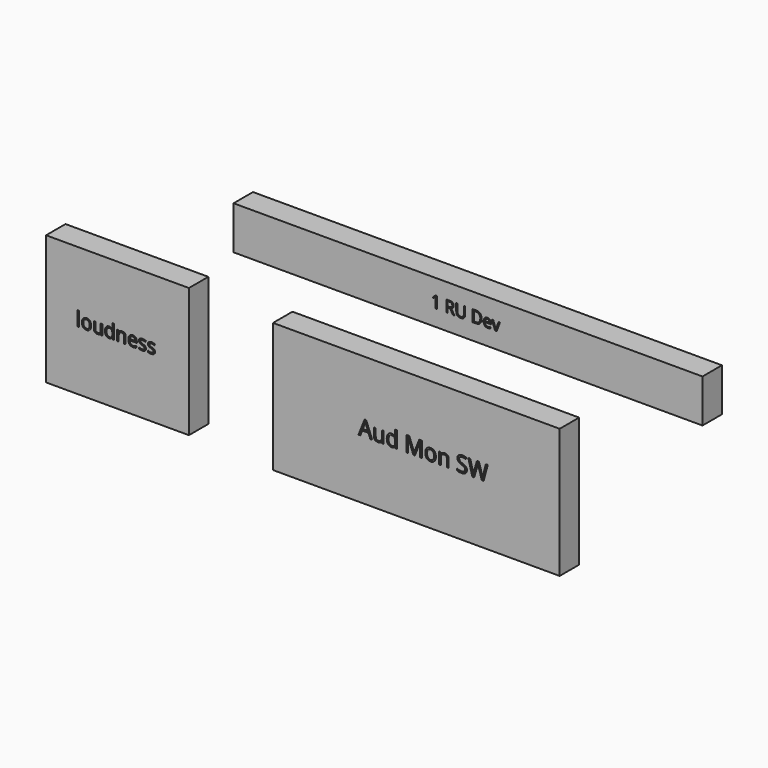
from build123d import *

# Parameters (mm, degrees)
F0_W           = 482.6
F0_H           = 44.45
F0_TEXT_SIZE   = 16.7372688237
F1_DEPTH       = 24
F0_W_2         = 147
F0_H_2         = 133.35
F0_W_3         = 1.5835024727
F0_H_3         = 14.8373266372
F0_TEXT_SIZE_2 = 19.5268127653
F2_DEPTH       = 24
F3_DEPTH       = 25
F0_W_4         = 295
F0_TEXT_SIZE_3 = 22.3163515329
F4_DEPTH       = 24
F5_DEPTH       = 25
F6_DEPTH       = 25


# Not quite as in the source:
# - Text() gives the source's letters only with a copy of the font that has no kerning and outlines rounded to 1/6400 em; it was checked with that copy


with BuildPart() as f1:
    # F0 (on Front) → F1 (new body)
    with BuildSketch(Plane.XZ):
        with Locations((-253.4153853834, 69.5086531699)):
            Rectangle(F0_W, F0_H)
        with BuildLine():
            Line((-285.4707886856, 75.858874375), (-285.4707886856, 63.9100335538))
            Line((-285.4707886856, 63.9100335538), (-286.794079002, 63.9100335538))
            Line((-286.794079002, 63.9100335538), (-286.794079002, 72.4251190679))
            add(Edge.make_bspline(
                [(-286.794079002, 72.4251190679), (-286.794079002, 73.4895047572), (-286.7286990457, 74.436206525)],
                knots=[0, 0, 0, 1, 1, 1], degree=2))
            add(Edge.make_bspline(
                [(-286.7286990457, 74.436206525), (-286.8986869321, 74.2636034403), (-287.1118255898, 74.0766167651)],
                knots=[0, 0, 0, 1, 1, 1], degree=2))
            add(Edge.make_bspline(
                [(-287.1118255898, 74.0766167651), (-287.3249642475, 73.88963009), (-289.0562254914, 72.4826534295)],
                knots=[0, 0, 0, 1, 1, 1], degree=2))
            Line((-289.0562254914, 72.4826534295), (-289.7754050112, 73.4136640078))
            Line((-289.7754050112, 73.4136640078), (-286.6136303225, 75.858874375))
            Line((-286.6136303225, 75.858874375), (-285.4707886856, 75.858874375))
        make_face(mode=Mode.SUBTRACT)
        with BuildLine():
            Line((-271.8691425681, 68.8789102359), (-274.3640417021, 68.8789102359))
            Line((-274.3640417021, 68.8789102359), (-274.3640417021, 63.9100335538))
            Line((-274.3640417021, 63.9100335538), (-275.7527119748, 63.9100335538))
            Line((-275.7527119748, 63.9100335538), (-275.7527119748, 75.858874375))
            Line((-275.7527119748, 75.858874375), (-272.475868563, 75.858874375))
            add(Edge.make_bspline(
                [(-272.475868563, 75.858874375), (-270.2764868316, 75.858874375), (-269.2264847327, 75.0167805373)],
                knots=[0, 0, 0, 1, 1, 1], degree=2))
            add(Edge.make_bspline(
                [(-269.2264847327, 75.0167805373), (-268.1764826339, 74.1746866996), (-268.1764826339, 72.4826534295)],
                knots=[0, 0, 0, 1, 1, 1], degree=2))
            add(Edge.make_bspline(
                [(-268.1764826339, 72.4826534295), (-268.1764826339, 70.1132838116), (-270.579849829, 69.2790355687)],
                knots=[0, 0, 0, 1, 1, 1], degree=2))
            Line((-270.579849829, 69.2790355687), (-267.3343887962, 63.9100335538))
            Line((-267.3343887962, 63.9100335538), (-268.9767332995, 63.9100335538))
            Line((-268.9767332995, 63.9100335538), (-271.8691425681, 68.8789102359))
        make_face(mode=Mode.SUBTRACT)
        with BuildLine():
            Line((-257.7732239806, 75.858874375), (-256.3845537079, 75.858874375))
            Line((-256.3845537079, 75.858874375), (-256.3845537079, 68.1283483371))
            add(Edge.make_bspline(
                [(-256.3845537079, 68.1283483371), (-256.3845537079, 66.0832633027), (-257.6189272837, 64.9142696833)],
                knots=[0, 0, 0, 1, 1, 1], degree=2))
            add(Edge.make_bspline(
                [(-257.6189272837, 64.9142696833), (-258.8533008594, 63.7452760639), (-261.0108394187, 63.7452760639)],
                knots=[0, 0, 0, 1, 1, 1], degree=2))
            add(Edge.make_bspline(
                [(-261.0108394187, 63.7452760639), (-263.168377978, 63.7452760639), (-264.3491399896, 64.9234228771)],
                knots=[0, 0, 0, 1, 1, 1], degree=2))
            add(Edge.make_bspline(
                [(-264.3491399896, 64.9234228771), (-265.5299020011, 66.1015696904), (-265.5299020011, 68.1597307161)],
                knots=[0, 0, 0, 1, 1, 1], degree=2))
            Line((-265.5299020011, 68.1597307161), (-265.5299020011, 75.858874375))
            Line((-265.5299020011, 75.858874375), (-264.1386165301, 75.858874375))
            Line((-264.1386165301, 75.858874375), (-264.1386165301, 68.0629683807))
            add(Edge.make_bspline(
                [(-264.1386165301, 68.0629683807), (-264.1386165301, 66.5670749796), (-263.3213670759, 65.7655167148)],
                knots=[0, 0, 0, 1, 1, 1], degree=2))
            add(Edge.make_bspline(
                [(-263.3213670759, 65.7655167148), (-262.5041176216, 64.9639584501), (-260.9193074798, 64.9639584501)],
                knots=[0, 0, 0, 1, 1, 1], degree=2))
            add(Edge.make_bspline(
                [(-260.9193074798, 64.9639584501), (-259.4077228892, 64.9639584501), (-258.5904734349, 65.7694395122)],
                knots=[0, 0, 0, 1, 1, 1], degree=2))
            add(Edge.make_bspline(
                [(-258.5904734349, 65.7694395122), (-257.7732239806, 66.5749205744), (-257.7732239806, 68.0786595702)],
                knots=[0, 0, 0, 1, 1, 1], degree=2))
            Line((-257.7732239806, 68.0786595702), (-257.7732239806, 75.858874375))
        make_face(mode=Mode.SUBTRACT)
        with BuildLine():
            add(Edge.make_bspline(
                [(-240.8803508608, 74.3145998062), (-239.336076292, 72.7703252374), (-239.336076292, 69.9982150885)],
                knots=[0, 0, 0, 1, 1, 1], degree=2))
            add(Edge.make_bspline(
                [(-239.336076292, 69.9982150885), (-239.336076292, 67.0404258635), (-240.9418080198, 65.4752297087)],
                knots=[0, 0, 0, 1, 1, 1], degree=2))
            add(Edge.make_bspline(
                [(-240.9418080198, 65.4752297087), (-242.5475397475, 63.9100335538), (-245.5628633341, 63.9100335538)],
                knots=[0, 0, 0, 1, 1, 1], degree=2))
            Line((-245.5628633341, 63.9100335538), (-248.8737043233, 63.9100335538))
            Line((-248.8737043233, 63.9100335538), (-248.8737043233, 75.858874375))
            Line((-248.8737043233, 75.858874375), (-245.2124267681, 75.858874375))
            add(Edge.make_bspline(
                [(-245.2124267681, 75.858874375), (-242.4246254296, 75.858874375), (-240.8803508608, 74.3145998062)],
                knots=[0, 0, 0, 1, 1, 1], degree=2))
        make_face(mode=Mode.SUBTRACT)
        with BuildLine():
            add(Edge.make_bspline(
                [(-231.542785496, 63.881266373), (-232.1835090681, 63.7452760639), (-233.0909828621, 63.7452760639)],
                knots=[0, 0, 0, 1, 1, 1], degree=2))
            add(Edge.make_bspline(
                [(-233.0909828621, 63.7452760639), (-235.0759183367, 63.7452760639), (-236.2252979692, 64.9561128553)],
                knots=[0, 0, 0, 1, 1, 1], degree=2))
            add(Edge.make_bspline(
                [(-236.2252979692, 64.9561128553), (-237.3746776017, 66.1669496468), (-237.3746776017, 68.3140274131)],
                knots=[0, 0, 0, 1, 1, 1], degree=2))
            add(Edge.make_bspline(
                [(-237.3746776017, 68.3140274131), (-237.3746776017, 70.4820267654), (-236.3076767142, 71.7569359141)],
                knots=[0, 0, 0, 1, 1, 1], degree=2))
            add(Edge.make_bspline(
                [(-236.3076767142, 71.7569359141), (-235.2406758267, 73.0318450628), (-233.4414194281, 73.0318450628)],
                knots=[0, 0, 0, 1, 1, 1], degree=2))
            add(Edge.make_bspline(
                [(-233.4414194281, 73.0318450628), (-231.759846951, 73.0318450628), (-230.7791476059, 71.9243086023)],
                knots=[0, 0, 0, 1, 1, 1], degree=2))
            add(Edge.make_bspline(
                [(-230.7791476059, 71.9243086023), (-229.7984482607, 70.8167721419), (-229.7984482607, 69.0018245538)],
                knots=[0, 0, 0, 1, 1, 1], degree=2))
            Line((-229.7984482607, 69.0018245538), (-229.7984482607, 68.1440395266))
            Line((-229.7984482607, 68.1440395266), (-235.9677009412, 68.1440395266))
            add(Edge.make_bspline(
                [(-235.9677009412, 68.1440395266), (-235.9258577692, 66.5670749796), (-235.1700654738, 65.7498255253)],
                knots=[0, 0, 0, 1, 1, 1], degree=2))
            add(Edge.make_bspline(
                [(-235.1700654738, 65.7498255253), (-234.4142731785, 64.932576071), (-233.0412940953, 64.932576071)],
                knots=[0, 0, 0, 1, 1, 1], degree=2))
            add(Edge.make_bspline(
                [(-233.0412940953, 64.932576071), (-231.595089461, 64.932576071), (-230.182882404, 65.5366868676)],
                knots=[0, 0, 0, 1, 1, 1], degree=2))
            Line((-230.182882404, 65.5366868676), (-230.182882404, 64.3258500762))
            add(Edge.make_bspline(
                [(-230.182882404, 64.3258500762), (-230.9020619238, 64.0172566822), (-231.542785496, 63.881266373)],
                knots=[0, 0, 0, 1, 1, 1], degree=2))
        make_face(mode=Mode.SUBTRACT)
        with BuildLine():
            Line((-223.9377889742, 63.9100335538), (-225.5225991159, 63.9100335538))
            Line((-225.5225991159, 63.9100335538), (-228.9223568457, 72.8670875728))
            Line((-228.9223568457, 72.8670875728), (-227.4683066167, 72.8670875728))
            Line((-227.4683066167, 72.8670875728), (-225.5382903054, 67.5556199195))
            add(Edge.make_bspline(
                [(-225.5382903054, 67.5556199195), (-224.884490742, 65.6909835646), (-224.7694220189, 65.1365615348)],
                knots=[0, 0, 0, 1, 1, 1], degree=2))
            Line((-224.7694220189, 65.1365615348), (-224.7040420625, 65.1365615348))
            add(Edge.make_bspline(
                [(-224.7040420625, 65.1365615348), (-224.6151253219, 65.5680692467), (-224.1365440415, 66.9292799377)],
                knots=[0, 0, 0, 1, 1, 1], degree=2))
            add(Edge.make_bspline(
                [(-224.1365440415, 66.9292799377), (-223.657962761, 68.2904906288), (-221.9920814734, 72.8670875728)],
                knots=[0, 0, 0, 1, 1, 1], degree=2))
            Line((-221.9920814734, 72.8670875728), (-220.5380312444, 72.8670875728))
            Line((-220.5380312444, 72.8670875728), (-223.9377889742, 63.9100335538))
        make_face(mode=Mode.SUBTRACT)
        with BuildLine():
            add(Edge.make_bspline(
                [(-242.057190075, 66.3330147359), (-240.8058177106, 67.5556199195), (-240.8058177106, 69.9485263216)],
                knots=[0, 0, 0, 1, 1, 1], degree=2))
            add(Edge.make_bspline(
                [(-240.8058177106, 69.9485263216), (-240.8058177106, 72.2865135605), (-241.9787341274, 73.4711983694)],
                knots=[0, 0, 0, 1, 1, 1], degree=2))
            add(Edge.make_bspline(
                [(-241.9787341274, 73.4711983694), (-243.1516505442, 74.6558831783), (-245.4661009987, 74.6558831783)],
                knots=[0, 0, 0, 1, 1, 1], degree=2))
            Line((-245.4661009987, 74.6558831783), (-247.4850340505, 74.6558831783))
            Line((-247.4850340505, 74.6558831783), (-247.4850340505, 65.1104095523))
            Line((-247.4850340505, 65.1104095523), (-245.7930007804, 65.1104095523))
            add(Edge.make_bspline(
                [(-245.7930007804, 65.1104095523), (-243.3085624394, 65.1104095523), (-242.057190075, 66.3330147359)],
                knots=[0, 0, 0, 1, 1, 1], degree=2))
        make_face()
        with BuildLine():
            Line((-274.3640417021, 74.6401919888), (-274.3640417021, 70.0714406396))
            Line((-274.3640417021, 70.0714406396), (-272.4575621752, 70.0714406396))
            add(Edge.make_bspline(
                [(-272.4575621752, 70.0714406396), (-270.9878207566, 70.0714406396), (-270.301331215, 70.6559374493)],
                knots=[0, 0, 0, 1, 1, 1], degree=2))
            add(Edge.make_bspline(
                [(-270.301331215, 70.6559374493), (-269.6148416734, 71.240434259), (-269.6148416734, 72.4094278784)],
                knots=[0, 0, 0, 1, 1, 1], degree=2))
            add(Edge.make_bspline(
                [(-269.6148416734, 72.4094278784), (-269.6148416734, 73.5941126873), (-270.3130996071, 74.1171523381)],
                knots=[0, 0, 0, 1, 1, 1], degree=2))
            add(Edge.make_bspline(
                [(-270.3130996071, 74.1171523381), (-271.0113575409, 74.6401919888), (-272.5569397088, 74.6401919888)],
                knots=[0, 0, 0, 1, 1, 1], degree=2))
            Line((-272.5569397088, 74.6401919888), (-274.3640417021, 74.6401919888))
        make_face()
        with Locations((-291.3131415844, 63.9100335538)):
            Text('1 RU Dev', F0_TEXT_SIZE, font='Open Sans', text_align=(TextAlign.LEFT, TextAlign.BOTTOM))
        with BuildLine():
            add(Edge.make_bspline(
                [(-231.8239193082, 71.2116670782), (-232.3953401267, 71.8942338224), (-233.4597258159, 71.8942338224)],
                knots=[0, 0, 0, 1, 1, 1], degree=2))
            add(Edge.make_bspline(
                [(-233.4597258159, 71.8942338224), (-234.5371874964, 71.8942338224), (-235.1792186677, 71.1920530913)],
                knots=[0, 0, 0, 1, 1, 1], degree=2))
            add(Edge.make_bspline(
                [(-235.1792186677, 71.1920530913), (-235.821249839, 70.4898723602), (-235.9363185622, 69.2476531897)],
                knots=[0, 0, 0, 1, 1, 1], degree=2))
            Line((-235.9363185622, 69.2476531897), (-231.2524984898, 69.2476531897))
            add(Edge.make_bspline(
                [(-231.2524984898, 69.2476531897), (-231.2524984898, 70.529100334), (-231.8239193082, 71.2116670782)],
                knots=[0, 0, 0, 1, 1, 1], degree=2))
        make_face()
    extrude(amount=F1_DEPTH)

    # F0 (on Front) → F6 (join)
    with BuildSketch(Plane.XZ):
        with Locations((-253.4153853834, 69.5086531699)):
            Rectangle(F0_W, F0_H)
        with BuildLine():
            Line((-285.4707886856, 75.858874375), (-285.4707886856, 63.9100335538))
            Line((-285.4707886856, 63.9100335538), (-286.794079002, 63.9100335538))
            Line((-286.794079002, 63.9100335538), (-286.794079002, 72.4251190679))
            add(Edge.make_bspline(
                [(-286.794079002, 72.4251190679), (-286.794079002, 73.4895047572), (-286.7286990457, 74.436206525)],
                knots=[0, 0, 0, 1, 1, 1], degree=2))
            add(Edge.make_bspline(
                [(-286.7286990457, 74.436206525), (-286.8986869321, 74.2636034403), (-287.1118255898, 74.0766167651)],
                knots=[0, 0, 0, 1, 1, 1], degree=2))
            add(Edge.make_bspline(
                [(-287.1118255898, 74.0766167651), (-287.3249642475, 73.88963009), (-289.0562254914, 72.4826534295)],
                knots=[0, 0, 0, 1, 1, 1], degree=2))
            Line((-289.0562254914, 72.4826534295), (-289.7754050112, 73.4136640078))
            Line((-289.7754050112, 73.4136640078), (-286.6136303225, 75.858874375))
            Line((-286.6136303225, 75.858874375), (-285.4707886856, 75.858874375))
        make_face(mode=Mode.SUBTRACT)
        with BuildLine():
            Line((-271.8691425681, 68.8789102359), (-274.3640417021, 68.8789102359))
            Line((-274.3640417021, 68.8789102359), (-274.3640417021, 63.9100335538))
            Line((-274.3640417021, 63.9100335538), (-275.7527119748, 63.9100335538))
            Line((-275.7527119748, 63.9100335538), (-275.7527119748, 75.858874375))
            Line((-275.7527119748, 75.858874375), (-272.475868563, 75.858874375))
            add(Edge.make_bspline(
                [(-272.475868563, 75.858874375), (-270.2764868316, 75.858874375), (-269.2264847327, 75.0167805373)],
                knots=[0, 0, 0, 1, 1, 1], degree=2))
            add(Edge.make_bspline(
                [(-269.2264847327, 75.0167805373), (-268.1764826339, 74.1746866996), (-268.1764826339, 72.4826534295)],
                knots=[0, 0, 0, 1, 1, 1], degree=2))
            add(Edge.make_bspline(
                [(-268.1764826339, 72.4826534295), (-268.1764826339, 70.1132838116), (-270.579849829, 69.2790355687)],
                knots=[0, 0, 0, 1, 1, 1], degree=2))
            Line((-270.579849829, 69.2790355687), (-267.3343887962, 63.9100335538))
            Line((-267.3343887962, 63.9100335538), (-268.9767332995, 63.9100335538))
            Line((-268.9767332995, 63.9100335538), (-271.8691425681, 68.8789102359))
        make_face(mode=Mode.SUBTRACT)
        with BuildLine():
            Line((-257.7732239806, 75.858874375), (-256.3845537079, 75.858874375))
            Line((-256.3845537079, 75.858874375), (-256.3845537079, 68.1283483371))
            add(Edge.make_bspline(
                [(-256.3845537079, 68.1283483371), (-256.3845537079, 66.0832633027), (-257.6189272837, 64.9142696833)],
                knots=[0, 0, 0, 1, 1, 1], degree=2))
            add(Edge.make_bspline(
                [(-257.6189272837, 64.9142696833), (-258.8533008594, 63.7452760639), (-261.0108394187, 63.7452760639)],
                knots=[0, 0, 0, 1, 1, 1], degree=2))
            add(Edge.make_bspline(
                [(-261.0108394187, 63.7452760639), (-263.168377978, 63.7452760639), (-264.3491399896, 64.9234228771)],
                knots=[0, 0, 0, 1, 1, 1], degree=2))
            add(Edge.make_bspline(
                [(-264.3491399896, 64.9234228771), (-265.5299020011, 66.1015696904), (-265.5299020011, 68.1597307161)],
                knots=[0, 0, 0, 1, 1, 1], degree=2))
            Line((-265.5299020011, 68.1597307161), (-265.5299020011, 75.858874375))
            Line((-265.5299020011, 75.858874375), (-264.1386165301, 75.858874375))
            Line((-264.1386165301, 75.858874375), (-264.1386165301, 68.0629683807))
            add(Edge.make_bspline(
                [(-264.1386165301, 68.0629683807), (-264.1386165301, 66.5670749796), (-263.3213670759, 65.7655167148)],
                knots=[0, 0, 0, 1, 1, 1], degree=2))
            add(Edge.make_bspline(
                [(-263.3213670759, 65.7655167148), (-262.5041176216, 64.9639584501), (-260.9193074798, 64.9639584501)],
                knots=[0, 0, 0, 1, 1, 1], degree=2))
            add(Edge.make_bspline(
                [(-260.9193074798, 64.9639584501), (-259.4077228892, 64.9639584501), (-258.5904734349, 65.7694395122)],
                knots=[0, 0, 0, 1, 1, 1], degree=2))
            add(Edge.make_bspline(
                [(-258.5904734349, 65.7694395122), (-257.7732239806, 66.5749205744), (-257.7732239806, 68.0786595702)],
                knots=[0, 0, 0, 1, 1, 1], degree=2))
            Line((-257.7732239806, 68.0786595702), (-257.7732239806, 75.858874375))
        make_face(mode=Mode.SUBTRACT)
        with BuildLine():
            add(Edge.make_bspline(
                [(-240.8803508608, 74.3145998062), (-239.336076292, 72.7703252374), (-239.336076292, 69.9982150885)],
                knots=[0, 0, 0, 1, 1, 1], degree=2))
            add(Edge.make_bspline(
                [(-239.336076292, 69.9982150885), (-239.336076292, 67.0404258635), (-240.9418080198, 65.4752297087)],
                knots=[0, 0, 0, 1, 1, 1], degree=2))
            add(Edge.make_bspline(
                [(-240.9418080198, 65.4752297087), (-242.5475397475, 63.9100335538), (-245.5628633341, 63.9100335538)],
                knots=[0, 0, 0, 1, 1, 1], degree=2))
            Line((-245.5628633341, 63.9100335538), (-248.8737043233, 63.9100335538))
            Line((-248.8737043233, 63.9100335538), (-248.8737043233, 75.858874375))
            Line((-248.8737043233, 75.858874375), (-245.2124267681, 75.858874375))
            add(Edge.make_bspline(
                [(-245.2124267681, 75.858874375), (-242.4246254296, 75.858874375), (-240.8803508608, 74.3145998062)],
                knots=[0, 0, 0, 1, 1, 1], degree=2))
        make_face(mode=Mode.SUBTRACT)
        with BuildLine():
            add(Edge.make_bspline(
                [(-231.542785496, 63.881266373), (-232.1835090681, 63.7452760639), (-233.0909828621, 63.7452760639)],
                knots=[0, 0, 0, 1, 1, 1], degree=2))
            add(Edge.make_bspline(
                [(-233.0909828621, 63.7452760639), (-235.0759183367, 63.7452760639), (-236.2252979692, 64.9561128553)],
                knots=[0, 0, 0, 1, 1, 1], degree=2))
            add(Edge.make_bspline(
                [(-236.2252979692, 64.9561128553), (-237.3746776017, 66.1669496468), (-237.3746776017, 68.3140274131)],
                knots=[0, 0, 0, 1, 1, 1], degree=2))
            add(Edge.make_bspline(
                [(-237.3746776017, 68.3140274131), (-237.3746776017, 70.4820267654), (-236.3076767142, 71.7569359141)],
                knots=[0, 0, 0, 1, 1, 1], degree=2))
            add(Edge.make_bspline(
                [(-236.3076767142, 71.7569359141), (-235.2406758267, 73.0318450628), (-233.4414194281, 73.0318450628)],
                knots=[0, 0, 0, 1, 1, 1], degree=2))
            add(Edge.make_bspline(
                [(-233.4414194281, 73.0318450628), (-231.759846951, 73.0318450628), (-230.7791476059, 71.9243086023)],
                knots=[0, 0, 0, 1, 1, 1], degree=2))
            add(Edge.make_bspline(
                [(-230.7791476059, 71.9243086023), (-229.7984482607, 70.8167721419), (-229.7984482607, 69.0018245538)],
                knots=[0, 0, 0, 1, 1, 1], degree=2))
            Line((-229.7984482607, 69.0018245538), (-229.7984482607, 68.1440395266))
            Line((-229.7984482607, 68.1440395266), (-235.9677009412, 68.1440395266))
            add(Edge.make_bspline(
                [(-235.9677009412, 68.1440395266), (-235.9258577692, 66.5670749796), (-235.1700654738, 65.7498255253)],
                knots=[0, 0, 0, 1, 1, 1], degree=2))
            add(Edge.make_bspline(
                [(-235.1700654738, 65.7498255253), (-234.4142731785, 64.932576071), (-233.0412940953, 64.932576071)],
                knots=[0, 0, 0, 1, 1, 1], degree=2))
            add(Edge.make_bspline(
                [(-233.0412940953, 64.932576071), (-231.595089461, 64.932576071), (-230.182882404, 65.5366868676)],
                knots=[0, 0, 0, 1, 1, 1], degree=2))
            Line((-230.182882404, 65.5366868676), (-230.182882404, 64.3258500762))
            add(Edge.make_bspline(
                [(-230.182882404, 64.3258500762), (-230.9020619238, 64.0172566822), (-231.542785496, 63.881266373)],
                knots=[0, 0, 0, 1, 1, 1], degree=2))
        make_face(mode=Mode.SUBTRACT)
        with BuildLine():
            Line((-223.9377889742, 63.9100335538), (-225.5225991159, 63.9100335538))
            Line((-225.5225991159, 63.9100335538), (-228.9223568457, 72.8670875728))
            Line((-228.9223568457, 72.8670875728), (-227.4683066167, 72.8670875728))
            Line((-227.4683066167, 72.8670875728), (-225.5382903054, 67.5556199195))
            add(Edge.make_bspline(
                [(-225.5382903054, 67.5556199195), (-224.884490742, 65.6909835646), (-224.7694220189, 65.1365615348)],
                knots=[0, 0, 0, 1, 1, 1], degree=2))
            Line((-224.7694220189, 65.1365615348), (-224.7040420625, 65.1365615348))
            add(Edge.make_bspline(
                [(-224.7040420625, 65.1365615348), (-224.6151253219, 65.5680692467), (-224.1365440415, 66.9292799377)],
                knots=[0, 0, 0, 1, 1, 1], degree=2))
            add(Edge.make_bspline(
                [(-224.1365440415, 66.9292799377), (-223.657962761, 68.2904906288), (-221.9920814734, 72.8670875728)],
                knots=[0, 0, 0, 1, 1, 1], degree=2))
            Line((-221.9920814734, 72.8670875728), (-220.5380312444, 72.8670875728))
            Line((-220.5380312444, 72.8670875728), (-223.9377889742, 63.9100335538))
        make_face(mode=Mode.SUBTRACT)
        with BuildLine():
            add(Edge.make_bspline(
                [(-242.057190075, 66.3330147359), (-240.8058177106, 67.5556199195), (-240.8058177106, 69.9485263216)],
                knots=[0, 0, 0, 1, 1, 1], degree=2))
            add(Edge.make_bspline(
                [(-240.8058177106, 69.9485263216), (-240.8058177106, 72.2865135605), (-241.9787341274, 73.4711983694)],
                knots=[0, 0, 0, 1, 1, 1], degree=2))
            add(Edge.make_bspline(
                [(-241.9787341274, 73.4711983694), (-243.1516505442, 74.6558831783), (-245.4661009987, 74.6558831783)],
                knots=[0, 0, 0, 1, 1, 1], degree=2))
            Line((-245.4661009987, 74.6558831783), (-247.4850340505, 74.6558831783))
            Line((-247.4850340505, 74.6558831783), (-247.4850340505, 65.1104095523))
            Line((-247.4850340505, 65.1104095523), (-245.7930007804, 65.1104095523))
            add(Edge.make_bspline(
                [(-245.7930007804, 65.1104095523), (-243.3085624394, 65.1104095523), (-242.057190075, 66.3330147359)],
                knots=[0, 0, 0, 1, 1, 1], degree=2))
        make_face()
        with BuildLine():
            Line((-274.3640417021, 74.6401919888), (-274.3640417021, 70.0714406396))
            Line((-274.3640417021, 70.0714406396), (-272.4575621752, 70.0714406396))
            add(Edge.make_bspline(
                [(-272.4575621752, 70.0714406396), (-270.9878207566, 70.0714406396), (-270.301331215, 70.6559374493)],
                knots=[0, 0, 0, 1, 1, 1], degree=2))
            add(Edge.make_bspline(
                [(-270.301331215, 70.6559374493), (-269.6148416734, 71.240434259), (-269.6148416734, 72.4094278784)],
                knots=[0, 0, 0, 1, 1, 1], degree=2))
            add(Edge.make_bspline(
                [(-269.6148416734, 72.4094278784), (-269.6148416734, 73.5941126873), (-270.3130996071, 74.1171523381)],
                knots=[0, 0, 0, 1, 1, 1], degree=2))
            add(Edge.make_bspline(
                [(-270.3130996071, 74.1171523381), (-271.0113575409, 74.6401919888), (-272.5569397088, 74.6401919888)],
                knots=[0, 0, 0, 1, 1, 1], degree=2))
            Line((-272.5569397088, 74.6401919888), (-274.3640417021, 74.6401919888))
        make_face()
        with BuildLine():
            add(Edge.make_bspline(
                [(-231.8239193082, 71.2116670782), (-232.3953401267, 71.8942338224), (-233.4597258159, 71.8942338224)],
                knots=[0, 0, 0, 1, 1, 1], degree=2))
            add(Edge.make_bspline(
                [(-233.4597258159, 71.8942338224), (-234.5371874964, 71.8942338224), (-235.1792186677, 71.1920530913)],
                knots=[0, 0, 0, 1, 1, 1], degree=2))
            add(Edge.make_bspline(
                [(-235.1792186677, 71.1920530913), (-235.821249839, 70.4898723602), (-235.9363185622, 69.2476531897)],
                knots=[0, 0, 0, 1, 1, 1], degree=2))
            Line((-235.9363185622, 69.2476531897), (-231.2524984898, 69.2476531897))
            add(Edge.make_bspline(
                [(-231.2524984898, 69.2476531897), (-231.2524984898, 70.529100334), (-231.8239193082, 71.2116670782)],
                knots=[0, 0, 0, 1, 1, 1], degree=2))
        make_face()
    extrude(amount=F6_DEPTH)


with BuildPart() as f2:
    # F0 (on Front) → F2 (new body)
    with BuildSketch(Plane.XZ):
        with Locations((-614.1529307365, -66.675)):
            Rectangle(F0_W_2, F0_H_2)
        with BuildLine():
            add(Edge.make_bspline(
                [(-642.5105266325, -62.9817720554), (-641.218400819, -64.4417064161), (-641.218400819, -66.9283239792)],
                knots=[0, 0, 0, 1, 1, 1], degree=2))
            add(Edge.make_bspline(
                [(-641.218400819, -66.9283239792), (-641.218400819, -69.4851160256), (-642.5044245035, -70.9206418703)],
                knots=[0, 0, 0, 1, 1, 1], degree=2))
            add(Edge.make_bspline(
                [(-642.5044245035, -70.9206418703), (-643.790448188, -72.356167715), (-646.0604401719, -72.356167715)],
                knots=[0, 0, 0, 1, 1, 1], degree=2))
            add(Edge.make_bspline(
                [(-646.0604401719, -72.356167715), (-647.4639298394, -72.356167715), (-648.5501087995, -71.6971377842)],
                knots=[0, 0, 0, 1, 1, 1], degree=2))
            add(Edge.make_bspline(
                [(-648.5501087995, -71.6971377842), (-649.6362877596, -71.0381078534), (-650.2281942715, -69.8085288621)],
                knots=[0, 0, 0, 1, 1, 1], degree=2))
            add(Edge.make_bspline(
                [(-650.2281942715, -69.8085288621), (-650.8201007835, -68.5789498707), (-650.8201007835, -66.9283239792)],
                knots=[0, 0, 0, 1, 1, 1], degree=2))
            add(Edge.make_bspline(
                [(-650.8201007835, -66.9283239792), (-650.8201007835, -64.3745829972), (-649.5417047602, -62.948210346)],
                knots=[0, 0, 0, 1, 1, 1], degree=2))
            add(Edge.make_bspline(
                [(-649.5417047602, -62.948210346), (-648.263308737, -61.5218376948), (-645.993316753, -61.5218376948)],
                knots=[0, 0, 0, 1, 1, 1], degree=2))
            add(Edge.make_bspline(
                [(-645.993316753, -61.5218376948), (-643.8026524459, -61.5218376948), (-642.5105266325, -62.9817720554)],
                knots=[0, 0, 0, 1, 1, 1], degree=2))
        make_face(mode=Mode.SUBTRACT)
        with BuildLine():
            Line((-638.5548215152, -61.7140547579), (-636.9530126556, -61.7140547579))
            Line((-636.9530126556, -61.7140547579), (-636.9530126556, -68.4935200649))
            add(Edge.make_bspline(
                [(-636.9530126556, -68.4935200649), (-636.9530126556, -69.7719160881), (-636.3717848694, -70.400435374)],
                knots=[0, 0, 0, 1, 1, 1], degree=2))
            add(Edge.make_bspline(
                [(-636.3717848694, -70.400435374), (-635.7905570832, -71.0289546599), (-634.5518248984, -71.0289546599)],
                knots=[0, 0, 0, 1, 1, 1], degree=2))
            add(Edge.make_bspline(
                [(-634.5518248984, -71.0289546599), (-632.9103522003, -71.0289546599), (-632.1536882056, -70.1334672307)],
                knots=[0, 0, 0, 1, 1, 1], degree=2))
            add(Edge.make_bspline(
                [(-632.1536882056, -70.1334672307), (-631.397024211, -69.2379798016), (-631.397024211, -67.2059708482)],
                knots=[0, 0, 0, 1, 1, 1], degree=2))
            Line((-631.397024211, -67.2059708482), (-631.397024211, -61.7140547579))
            Line((-631.397024211, -61.7140547579), (-629.8135217383, -61.7140547579))
            Line((-629.8135217383, -61.7140547579), (-629.8135217383, -72.1639506519))
            Line((-629.8135217383, -72.1639506519), (-631.1193773419, -72.1639506519))
            Line((-631.1193773419, -72.1639506519), (-631.348207179, -70.7635120489))
            Line((-631.348207179, -70.7635120489), (-631.4336369849, -70.7635120489))
            add(Edge.make_bspline(
                [(-631.4336369849, -70.7635120489), (-631.9187562395, -71.535431366), (-632.7822074915, -71.9457995405)],
                knots=[0, 0, 0, 1, 1, 1], degree=2))
            add(Edge.make_bspline(
                [(-632.7822074915, -71.9457995405), (-633.6456587435, -72.356167715), (-634.753195155, -72.356167715)],
                knots=[0, 0, 0, 1, 1, 1], degree=2))
            add(Edge.make_bspline(
                [(-634.753195155, -72.356167715), (-636.6601104641, -72.356167715), (-637.6074659897, -71.4500015602)],
                knots=[0, 0, 0, 1, 1, 1], degree=2))
            add(Edge.make_bspline(
                [(-637.6074659897, -71.4500015602), (-638.5548215152, -70.5438354053), (-638.5548215152, -68.5514902903)],
                knots=[0, 0, 0, 1, 1, 1], degree=2))
            Line((-638.5548215152, -68.5514902903), (-638.5548215152, -61.7140547579))
        make_face(mode=Mode.SUBTRACT)
        with BuildLine():
            Line((-605.7558781985, -72.1639506519), (-607.3393806712, -72.1639506519))
            Line((-607.3393806712, -72.1639506519), (-607.3393806712, -65.4027917319))
            add(Edge.make_bspline(
                [(-607.3393806712, -65.4027917319), (-607.3393806712, -64.1274467732), (-607.9206084574, -63.497401955)],
                knots=[0, 0, 0, 1, 1, 1], degree=2))
            add(Edge.make_bspline(
                [(-607.9206084574, -63.497401955), (-608.5018362436, -62.8673571369), (-609.7436194929, -62.8673571369)],
                knots=[0, 0, 0, 1, 1, 1], degree=2))
            add(Edge.make_bspline(
                [(-609.7436194929, -62.8673571369), (-611.3820411265, -62.8673571369), (-612.1448072501, -63.7536913726)],
                knots=[0, 0, 0, 1, 1, 1], degree=2))
            add(Edge.make_bspline(
                [(-612.1448072501, -63.7536913726), (-612.9075733738, -64.6400256082), (-612.9075733738, -66.6811877551)],
                knots=[0, 0, 0, 1, 1, 1], degree=2))
            Line((-612.9075733738, -66.6811877551), (-612.9075733738, -72.1639506519))
            Line((-612.9075733738, -72.1639506519), (-614.4910758465, -72.1639506519))
            Line((-614.4910758465, -72.1639506519), (-614.4910758465, -61.7140547579))
            Line((-614.4910758465, -61.7140547579), (-613.2035266298, -61.7140547579))
            Line((-613.2035266298, -61.7140547579), (-612.9472372122, -63.1450040059))
            Line((-612.9472372122, -63.1450040059), (-612.8709605998, -63.1450040059))
            add(Edge.make_bspline(
                [(-612.8709605998, -63.1450040059), (-612.3827902807, -62.3730846888), (-611.5056092385, -61.9474611918)],
                knots=[0, 0, 0, 1, 1, 1], degree=2))
            add(Edge.make_bspline(
                [(-611.5056092385, -61.9474611918), (-610.6284281963, -61.5218376948), (-609.5514024297, -61.5218376948)],
                knots=[0, 0, 0, 1, 1, 1], degree=2))
            add(Edge.make_bspline(
                [(-609.5514024297, -61.5218376948), (-607.6627935076, -61.5218376948), (-606.709335853, -62.4325804464)],
                knots=[0, 0, 0, 1, 1, 1], degree=2))
            add(Edge.make_bspline(
                [(-606.709335853, -62.4325804464), (-605.7558781985, -63.343323198), (-605.7558781985, -65.347872571)],
                knots=[0, 0, 0, 1, 1, 1], degree=2))
            Line((-605.7558781985, -65.347872571), (-605.7558781985, -72.1639506519))
        make_face(mode=Mode.SUBTRACT)
        with Locations((-654.3852696454, -64.7452873333)):
            Rectangle(F0_W_3, F0_H_3, mode=Mode.SUBTRACT)
        with BuildLine():
            Line((-619.1347960072, -72.1639506519), (-619.3453194574, -70.7635120489))
            Line((-619.3453194574, -70.7635120489), (-619.4307492632, -70.7635120489))
            add(Edge.make_bspline(
                [(-619.4307492632, -70.7635120489), (-620.5260814168, -72.356167715), (-622.7106435949, -72.356167715)],
                knots=[0, 0, 0, 1, 1, 1], degree=2))
            add(Edge.make_bspline(
                [(-622.7106435949, -72.356167715), (-624.7609589352, -72.356167715), (-625.900531524, -70.9542035798)],
                knots=[0, 0, 0, 1, 1, 1], degree=2))
            add(Edge.make_bspline(
                [(-625.900531524, -70.9542035798), (-627.0401041127, -69.5522394445), (-627.0401041127, -66.9679878176)],
                knots=[0, 0, 0, 1, 1, 1], degree=2))
            add(Edge.make_bspline(
                [(-627.0401041127, -66.9679878176), (-627.0401041127, -64.3837361907), (-625.8959549272, -62.9527869427)],
                knots=[0, 0, 0, 1, 1, 1], degree=2))
            add(Edge.make_bspline(
                [(-625.8959549272, -62.9527869427), (-624.7518057418, -61.5218376948), (-622.7106435949, -61.5218376948)],
                knots=[0, 0, 0, 1, 1, 1], degree=2))
            add(Edge.make_bspline(
                [(-622.7106435949, -61.5218376948), (-620.5840516422, -61.5218376948), (-619.4490556502, -63.0687273935)],
                knots=[0, 0, 0, 1, 1, 1], degree=2))
            Line((-619.4490556502, -63.0687273935), (-619.3239620059, -63.0687273935))
            Line((-619.3239620059, -63.0687273935), (-619.3910854248, -62.3151144634))
            Line((-619.3910854248, -62.3151144634), (-619.4307492632, -61.5798079202))
            Line((-619.4307492632, -61.5798079202), (-619.4307492632, -57.3266240147))
            Line((-619.4307492632, -57.3266240147), (-617.8472467905, -57.3266240147))
            Line((-617.8472467905, -57.3266240147), (-617.8472467905, -72.1639506519))
            Line((-617.8472467905, -72.1639506519), (-619.1347960072, -72.1639506519))
        make_face(mode=Mode.SUBTRACT)
        with BuildLine():
            add(Edge.make_bspline(
                [(-596.2853740073, -72.1975123613), (-597.0328848085, -72.356167715), (-598.0916041881, -72.356167715)],
                knots=[0, 0, 0, 1, 1, 1], degree=2))
            add(Edge.make_bspline(
                [(-598.0916041881, -72.356167715), (-600.4073621395, -72.356167715), (-601.7483049848, -70.9435248541)],
                knots=[0, 0, 0, 1, 1, 1], degree=2))
            add(Edge.make_bspline(
                [(-601.7483049848, -70.9435248541), (-603.0892478302, -69.5308819931), (-603.0892478302, -67.025958043)],
                knots=[0, 0, 0, 1, 1, 1], degree=2))
            add(Edge.make_bspline(
                [(-603.0892478302, -67.025958043), (-603.0892478302, -64.496625577), (-601.8444135164, -63.0092316359)],
                knots=[0, 0, 0, 1, 1, 1], degree=2))
            add(Edge.make_bspline(
                [(-601.8444135164, -63.0092316359), (-600.5995792026, -61.5218376948), (-598.5004468304, -61.5218376948)],
                knots=[0, 0, 0, 1, 1, 1], degree=2))
            add(Edge.make_bspline(
                [(-598.5004468304, -61.5218376948), (-596.5386123603, -61.5218376948), (-595.3944631749, -62.8139635082)],
                knots=[0, 0, 0, 1, 1, 1], degree=2))
            add(Edge.make_bspline(
                [(-595.3944631749, -62.8139635082), (-594.2503139894, -64.1060893217), (-594.2503139894, -66.2235280809)],
                knots=[0, 0, 0, 1, 1, 1], degree=2))
            Line((-594.2503139894, -66.2235280809), (-594.2503139894, -67.2242772352))
            Line((-594.2503139894, -67.2242772352), (-601.4477751321, -67.2242772352))
            add(Edge.make_bspline(
                [(-601.4477751321, -67.2242772352), (-601.3989581002, -69.0640691254), (-600.5172004613, -70.0175267799)],
                knots=[0, 0, 0, 1, 1, 1], degree=2))
            add(Edge.make_bspline(
                [(-600.5172004613, -70.0175267799), (-599.6354428223, -70.9709844345), (-598.0336339627, -70.9709844345)],
                knots=[0, 0, 0, 1, 1, 1], degree=2))
            add(Edge.make_bspline(
                [(-598.0336339627, -70.9709844345), (-596.3463952972, -70.9709844345), (-594.6988204701, -70.2661885363)],
                knots=[0, 0, 0, 1, 1, 1], degree=2))
            Line((-594.6988204701, -70.2661885363), (-594.6988204701, -71.6788313972))
            add(Edge.make_bspline(
                [(-594.6988204701, -71.6788313972), (-595.5378632061, -72.0388570076), (-596.2853740073, -72.1975123613)],
                knots=[0, 0, 0, 1, 1, 1], degree=2))
        make_face(mode=Mode.SUBTRACT)
        with BuildLine():
            add(Edge.make_bspline(
                [(-585.463248245, -67.58735391), (-584.8103204432, -68.2738434213), (-584.8103204432, -69.3142564139)],
                knots=[0, 0, 0, 1, 1, 1], degree=2))
            add(Edge.make_bspline(
                [(-584.8103204432, -69.3142564139), (-584.8103204432, -70.7726652424), (-585.8964994032, -71.5644164787)],
                knots=[0, 0, 0, 1, 1, 1], degree=2))
            add(Edge.make_bspline(
                [(-585.8964994032, -71.5644164787), (-586.9826783633, -72.356167715), (-588.9475638978, -72.356167715)],
                knots=[0, 0, 0, 1, 1, 1], degree=2))
            add(Edge.make_bspline(
                [(-588.9475638978, -72.356167715), (-591.0253388186, -72.356167715), (-592.1877943911, -71.6971377842)],
                knots=[0, 0, 0, 1, 1, 1], degree=2))
            Line((-592.1877943911, -71.6971377842), (-592.1877943911, -70.2295757623))
            add(Edge.make_bspline(
                [(-592.1877943911, -70.2295757623), (-591.4341814609, -70.6109588241), (-590.5722557412, -70.8291099355)],
                knots=[0, 0, 0, 1, 1, 1], degree=2))
            add(Edge.make_bspline(
                [(-590.5722557412, -70.8291099355), (-589.7103300215, -71.0472610469), (-588.9079000594, -71.0472610469)],
                knots=[0, 0, 0, 1, 1, 1], degree=2))
            add(Edge.make_bspline(
                [(-588.9079000594, -71.0472610469), (-587.6691678746, -71.0472610469), (-587.0025102825, -70.6521481948)],
                knots=[0, 0, 0, 1, 1, 1], degree=2))
            add(Edge.make_bspline(
                [(-587.0025102825, -70.6521481948), (-586.3358526905, -70.2570353428), (-586.3358526905, -69.4454521872)],
                knots=[0, 0, 0, 1, 1, 1], degree=2))
            add(Edge.make_bspline(
                [(-586.3358526905, -69.4454521872), (-586.3358526905, -68.8352392883), (-586.863686848, -68.4019881301)],
                knots=[0, 0, 0, 1, 1, 1], degree=2))
            add(Edge.make_bspline(
                [(-586.863686848, -68.4019881301), (-587.3915210056, -67.9687369718), (-588.9292575109, -67.3768304599)],
                knots=[0, 0, 0, 1, 1, 1], degree=2))
            add(Edge.make_bspline(
                [(-588.9292575109, -67.3768304599), (-590.3876663393, -66.8337409798), (-591.0024558349, -66.4279494021)],
                knots=[0, 0, 0, 1, 1, 1], degree=2))
            add(Edge.make_bspline(
                [(-591.0024558349, -66.4279494021), (-591.6172453306, -66.0221578243), (-591.9177751833, -65.508053457)],
                knots=[0, 0, 0, 1, 1, 1], degree=2))
            add(Edge.make_bspline(
                [(-591.9177751833, -65.508053457), (-592.218305036, -64.9939490896), (-592.218305036, -64.2799999979)],
                knots=[0, 0, 0, 1, 1, 1], degree=2))
            add(Edge.make_bspline(
                [(-592.218305036, -64.2799999979), (-592.218305036, -63.0016039747), (-591.1778920434, -62.2617208347)],
                knots=[0, 0, 0, 1, 1, 1], degree=2))
            add(Edge.make_bspline(
                [(-591.1778920434, -62.2617208347), (-590.1374790507, -61.5218376948), (-588.3281978054, -61.5218376948)],
                knots=[0, 0, 0, 1, 1, 1], degree=2))
            add(Edge.make_bspline(
                [(-588.3281978054, -61.5218376948), (-586.6409591399, -61.5218376948), (-585.0269460223, -62.2083272061)],
                knots=[0, 0, 0, 1, 1, 1], degree=2))
            Line((-585.0269460223, -62.2083272061), (-585.5913929538, -63.4958764228))
            add(Edge.make_bspline(
                [(-585.5913929538, -63.4958764228), (-587.1626911685, -62.8490507499), (-588.4410871917, -62.8490507499)],
                knots=[0, 0, 0, 1, 1, 1], degree=2))
            add(Edge.make_bspline(
                [(-588.4410871917, -62.8490507499), (-589.5669299902, -62.8490507499), (-590.139004583, -63.201448699)],
                knots=[0, 0, 0, 1, 1, 1], degree=2))
            add(Edge.make_bspline(
                [(-590.139004583, -63.201448699), (-590.7110791757, -63.5538466482), (-590.7110791757, -64.1732127406)],
                knots=[0, 0, 0, 1, 1, 1], degree=2))
            add(Edge.make_bspline(
                [(-590.7110791757, -64.1732127406), (-590.7110791757, -64.5942596408), (-590.4959791288, -64.8886873646)],
                knots=[0, 0, 0, 1, 1, 1], degree=2))
            add(Edge.make_bspline(
                [(-590.4959791288, -64.8886873646), (-590.280879082, -65.1831150883), (-589.8049130208, -65.4500832316)],
                knots=[0, 0, 0, 1, 1, 1], degree=2))
            add(Edge.make_bspline(
                [(-589.8049130208, -65.4500832316), (-589.3289469596, -65.7170513748), (-587.974274324, -66.2235280809)],
                knots=[0, 0, 0, 1, 1, 1], degree=2))
            add(Edge.make_bspline(
                [(-587.974274324, -66.2235280809), (-586.1161760468, -66.9008643987), (-585.463248245, -67.58735391)],
                knots=[0, 0, 0, 1, 1, 1], degree=2))
        make_face(mode=Mode.SUBTRACT)
        with BuildLine():
            add(Edge.make_bspline(
                [(-576.148348343, -67.58735391), (-575.4954205412, -68.2738434213), (-575.4954205412, -69.3142564139)],
                knots=[0, 0, 0, 1, 1, 1], degree=2))
            add(Edge.make_bspline(
                [(-575.4954205412, -69.3142564139), (-575.4954205412, -70.7726652424), (-576.5815995013, -71.5644164787)],
                knots=[0, 0, 0, 1, 1, 1], degree=2))
            add(Edge.make_bspline(
                [(-576.5815995013, -71.5644164787), (-577.6677784613, -72.356167715), (-579.6326639959, -72.356167715)],
                knots=[0, 0, 0, 1, 1, 1], degree=2))
            add(Edge.make_bspline(
                [(-579.6326639959, -72.356167715), (-581.7104389167, -72.356167715), (-582.8728944891, -71.6971377842)],
                knots=[0, 0, 0, 1, 1, 1], degree=2))
            Line((-582.8728944891, -71.6971377842), (-582.8728944891, -70.2295757623))
            add(Edge.make_bspline(
                [(-582.8728944891, -70.2295757623), (-582.1192815589, -70.6109588241), (-581.2573558392, -70.8291099355)],
                knots=[0, 0, 0, 1, 1, 1], degree=2))
            add(Edge.make_bspline(
                [(-581.2573558392, -70.8291099355), (-580.3954301195, -71.0472610469), (-579.5930001574, -71.0472610469)],
                knots=[0, 0, 0, 1, 1, 1], degree=2))
            add(Edge.make_bspline(
                [(-579.5930001574, -71.0472610469), (-578.3542679726, -71.0472610469), (-577.6876103806, -70.6521481948)],
                knots=[0, 0, 0, 1, 1, 1], degree=2))
            add(Edge.make_bspline(
                [(-577.6876103806, -70.6521481948), (-577.0209527885, -70.2570353428), (-577.0209527885, -69.4454521872)],
                knots=[0, 0, 0, 1, 1, 1], degree=2))
            add(Edge.make_bspline(
                [(-577.0209527885, -69.4454521872), (-577.0209527885, -68.8352392883), (-577.5487869461, -68.4019881301)],
                knots=[0, 0, 0, 1, 1, 1], degree=2))
            add(Edge.make_bspline(
                [(-577.5487869461, -68.4019881301), (-578.0766211036, -67.9687369718), (-579.6143576089, -67.3768304599)],
                knots=[0, 0, 0, 1, 1, 1], degree=2))
            add(Edge.make_bspline(
                [(-579.6143576089, -67.3768304599), (-581.0727664373, -66.8337409798), (-581.687555933, -66.4279494021)],
                knots=[0, 0, 0, 1, 1, 1], degree=2))
            add(Edge.make_bspline(
                [(-581.687555933, -66.4279494021), (-582.3023454286, -66.0221578243), (-582.6028752813, -65.508053457)],
                knots=[0, 0, 0, 1, 1, 1], degree=2))
            add(Edge.make_bspline(
                [(-582.6028752813, -65.508053457), (-582.903405134, -64.9939490896), (-582.903405134, -64.2799999979)],
                knots=[0, 0, 0, 1, 1, 1], degree=2))
            add(Edge.make_bspline(
                [(-582.903405134, -64.2799999979), (-582.903405134, -63.0016039747), (-581.8629921414, -62.2617208347)],
                knots=[0, 0, 0, 1, 1, 1], degree=2))
            add(Edge.make_bspline(
                [(-581.8629921414, -62.2617208347), (-580.8225791487, -61.5218376948), (-579.0132979035, -61.5218376948)],
                knots=[0, 0, 0, 1, 1, 1], degree=2))
            add(Edge.make_bspline(
                [(-579.0132979035, -61.5218376948), (-577.326059238, -61.5218376948), (-575.7120461203, -62.2083272061)],
                knots=[0, 0, 0, 1, 1, 1], degree=2))
            Line((-575.7120461203, -62.2083272061), (-576.2764930518, -63.4958764228))
            add(Edge.make_bspline(
                [(-576.2764930518, -63.4958764228), (-577.8477912665, -62.8490507499), (-579.1261872898, -62.8490507499)],
                knots=[0, 0, 0, 1, 1, 1], degree=2))
            add(Edge.make_bspline(
                [(-579.1261872898, -62.8490507499), (-580.2520300883, -62.8490507499), (-580.824104681, -63.201448699)],
                knots=[0, 0, 0, 1, 1, 1], degree=2))
            add(Edge.make_bspline(
                [(-580.824104681, -63.201448699), (-581.3961792737, -63.5538466482), (-581.3961792737, -64.1732127406)],
                knots=[0, 0, 0, 1, 1, 1], degree=2))
            add(Edge.make_bspline(
                [(-581.3961792737, -64.1732127406), (-581.3961792737, -64.5942596408), (-581.1810792269, -64.8886873646)],
                knots=[0, 0, 0, 1, 1, 1], degree=2))
            add(Edge.make_bspline(
                [(-581.1810792269, -64.8886873646), (-580.96597918, -65.1831150883), (-580.4900131188, -65.4500832316)],
                knots=[0, 0, 0, 1, 1, 1], degree=2))
            add(Edge.make_bspline(
                [(-580.4900131188, -65.4500832316), (-580.0140470577, -65.7170513748), (-578.6593744221, -66.2235280809)],
                knots=[0, 0, 0, 1, 1, 1], degree=2))
            add(Edge.make_bspline(
                [(-578.6593744221, -66.2235280809), (-576.8012761449, -66.9008643987), (-576.148348343, -67.58735391)],
                knots=[0, 0, 0, 1, 1, 1], degree=2))
        make_face(mode=Mode.SUBTRACT)
        with BuildLine():
            add(Edge.make_bspline(
                [(-648.386876849, -63.8879382103), (-649.1786280854, -64.9085192838), (-649.1786280854, -66.9283239792)],
                knots=[0, 0, 0, 1, 1, 1], degree=2))
            add(Edge.make_bspline(
                [(-649.1786280854, -66.9283239792), (-649.1786280854, -68.9328733521), (-648.3777236556, -69.980914006)],
                knots=[0, 0, 0, 1, 1, 1], degree=2))
            add(Edge.make_bspline(
                [(-648.3777236556, -69.980914006), (-647.5768192257, -71.0289546599), (-646.023827398, -71.0289546599)],
                knots=[0, 0, 0, 1, 1, 1], degree=2))
            add(Edge.make_bspline(
                [(-646.023827398, -71.0289546599), (-644.4677845058, -71.0289546599), (-643.6623034792, -69.9854906028)],
                knots=[0, 0, 0, 1, 1, 1], degree=2))
            add(Edge.make_bspline(
                [(-643.6623034792, -69.9854906028), (-642.8568224526, -68.9420265456), (-642.8568224526, -66.9283239792)],
                knots=[0, 0, 0, 1, 1, 1], degree=2))
            add(Edge.make_bspline(
                [(-642.8568224526, -66.9283239792), (-642.8568224526, -64.9359788642), (-643.6623034792, -63.9016680006)],
                knots=[0, 0, 0, 1, 1, 1], degree=2))
            add(Edge.make_bspline(
                [(-643.6623034792, -63.9016680006), (-644.4677845058, -62.8673571369), (-646.042133785, -62.8673571369)],
                knots=[0, 0, 0, 1, 1, 1], degree=2))
            add(Edge.make_bspline(
                [(-646.042133785, -62.8673571369), (-647.5951256127, -62.8673571369), (-648.386876849, -63.8879382103)],
                knots=[0, 0, 0, 1, 1, 1], degree=2))
        make_face()
        with BuildLine():
            add(Edge.make_bspline(
                [(-624.6648504037, -70.0083735865), (-623.9310693927, -71.0289546599), (-622.5092733382, -71.0289546599)],
                knots=[0, 0, 0, 1, 1, 1], degree=2))
            add(Edge.make_bspline(
                [(-622.5092733382, -71.0289546599), (-620.8891580916, -71.0289546599), (-620.1599536774, -70.147197021)],
                knots=[0, 0, 0, 1, 1, 1], degree=2))
            add(Edge.make_bspline(
                [(-620.1599536774, -70.147197021), (-619.4307492632, -69.265439382), (-619.4307492632, -67.3005538475)],
                knots=[0, 0, 0, 1, 1, 1], degree=2))
            Line((-619.4307492632, -67.3005538475), (-619.4307492632, -66.9679878176))
            add(Edge.make_bspline(
                [(-619.4307492632, -66.9679878176), (-619.4307492632, -64.7468128656), (-620.1691068709, -63.7979318077)],
                knots=[0, 0, 0, 1, 1, 1], degree=2))
            add(Edge.make_bspline(
                [(-620.1691068709, -63.7979318077), (-620.9074644786, -62.8490507499), (-622.5275797252, -62.8490507499)],
                knots=[0, 0, 0, 1, 1, 1], degree=2))
            add(Edge.make_bspline(
                [(-622.5275797252, -62.8490507499), (-623.9219161992, -62.8490507499), (-624.6602738069, -63.9306531133)],
                knots=[0, 0, 0, 1, 1, 1], degree=2))
            add(Edge.make_bspline(
                [(-624.6602738069, -63.9306531133), (-625.3986314146, -65.0122554766), (-625.3986314146, -66.9862942046)],
                knots=[0, 0, 0, 1, 1, 1], degree=2))
            add(Edge.make_bspline(
                [(-625.3986314146, -66.9862942046), (-625.3986314146, -68.987792513), (-624.6648504037, -70.0083735865)],
                knots=[0, 0, 0, 1, 1, 1], degree=2))
        make_face()
        with Locations((-656.8551063538, -72.1639506519)):
            Text('loudness', F0_TEXT_SIZE_2, font='Open Sans', text_align=(TextAlign.LEFT, TextAlign.BOTTOM))
        with BuildLine():
            add(Edge.make_bspline(
                [(-596.6133634405, -63.645378583), (-597.2800210325, -62.8490507499), (-598.5218042818, -62.8490507499)],
                knots=[0, 0, 0, 1, 1, 1], degree=2))
            add(Edge.make_bspline(
                [(-598.5218042818, -62.8490507499), (-599.7788428536, -62.8490507499), (-600.527879187, -63.6682615667)],
                knots=[0, 0, 0, 1, 1, 1], degree=2))
            add(Edge.make_bspline(
                [(-600.527879187, -63.6682615667), (-601.2769155204, -64.4874723835), (-601.4111623582, -65.9367280184)],
                knots=[0, 0, 0, 1, 1, 1], degree=2))
            Line((-601.4111623582, -65.9367280184), (-595.9467058484, -65.9367280184))
            add(Edge.make_bspline(
                [(-595.9467058484, -65.9367280184), (-595.9467058484, -64.4417064161), (-596.6133634405, -63.645378583)],
                knots=[0, 0, 0, 1, 1, 1], degree=2))
        make_face()
    extrude(amount=F2_DEPTH)

    # F0 (on Front) → F3 (join)
    with BuildSketch(Plane.XZ):
        with Locations((-614.1529307365, -66.675)):
            Rectangle(F0_W_2, F0_H_2)
        with BuildLine():
            add(Edge.make_bspline(
                [(-642.5105266325, -62.9817720554), (-641.218400819, -64.4417064161), (-641.218400819, -66.9283239792)],
                knots=[0, 0, 0, 1, 1, 1], degree=2))
            add(Edge.make_bspline(
                [(-641.218400819, -66.9283239792), (-641.218400819, -69.4851160256), (-642.5044245035, -70.9206418703)],
                knots=[0, 0, 0, 1, 1, 1], degree=2))
            add(Edge.make_bspline(
                [(-642.5044245035, -70.9206418703), (-643.790448188, -72.356167715), (-646.0604401719, -72.356167715)],
                knots=[0, 0, 0, 1, 1, 1], degree=2))
            add(Edge.make_bspline(
                [(-646.0604401719, -72.356167715), (-647.4639298394, -72.356167715), (-648.5501087995, -71.6971377842)],
                knots=[0, 0, 0, 1, 1, 1], degree=2))
            add(Edge.make_bspline(
                [(-648.5501087995, -71.6971377842), (-649.6362877596, -71.0381078534), (-650.2281942715, -69.8085288621)],
                knots=[0, 0, 0, 1, 1, 1], degree=2))
            add(Edge.make_bspline(
                [(-650.2281942715, -69.8085288621), (-650.8201007835, -68.5789498707), (-650.8201007835, -66.9283239792)],
                knots=[0, 0, 0, 1, 1, 1], degree=2))
            add(Edge.make_bspline(
                [(-650.8201007835, -66.9283239792), (-650.8201007835, -64.3745829972), (-649.5417047602, -62.948210346)],
                knots=[0, 0, 0, 1, 1, 1], degree=2))
            add(Edge.make_bspline(
                [(-649.5417047602, -62.948210346), (-648.263308737, -61.5218376948), (-645.993316753, -61.5218376948)],
                knots=[0, 0, 0, 1, 1, 1], degree=2))
            add(Edge.make_bspline(
                [(-645.993316753, -61.5218376948), (-643.8026524459, -61.5218376948), (-642.5105266325, -62.9817720554)],
                knots=[0, 0, 0, 1, 1, 1], degree=2))
        make_face(mode=Mode.SUBTRACT)
        with BuildLine():
            Line((-638.5548215152, -61.7140547579), (-636.9530126556, -61.7140547579))
            Line((-636.9530126556, -61.7140547579), (-636.9530126556, -68.4935200649))
            add(Edge.make_bspline(
                [(-636.9530126556, -68.4935200649), (-636.9530126556, -69.7719160881), (-636.3717848694, -70.400435374)],
                knots=[0, 0, 0, 1, 1, 1], degree=2))
            add(Edge.make_bspline(
                [(-636.3717848694, -70.400435374), (-635.7905570832, -71.0289546599), (-634.5518248984, -71.0289546599)],
                knots=[0, 0, 0, 1, 1, 1], degree=2))
            add(Edge.make_bspline(
                [(-634.5518248984, -71.0289546599), (-632.9103522003, -71.0289546599), (-632.1536882056, -70.1334672307)],
                knots=[0, 0, 0, 1, 1, 1], degree=2))
            add(Edge.make_bspline(
                [(-632.1536882056, -70.1334672307), (-631.397024211, -69.2379798016), (-631.397024211, -67.2059708482)],
                knots=[0, 0, 0, 1, 1, 1], degree=2))
            Line((-631.397024211, -67.2059708482), (-631.397024211, -61.7140547579))
            Line((-631.397024211, -61.7140547579), (-629.8135217383, -61.7140547579))
            Line((-629.8135217383, -61.7140547579), (-629.8135217383, -72.1639506519))
            Line((-629.8135217383, -72.1639506519), (-631.1193773419, -72.1639506519))
            Line((-631.1193773419, -72.1639506519), (-631.348207179, -70.7635120489))
            Line((-631.348207179, -70.7635120489), (-631.4336369849, -70.7635120489))
            add(Edge.make_bspline(
                [(-631.4336369849, -70.7635120489), (-631.9187562395, -71.535431366), (-632.7822074915, -71.9457995405)],
                knots=[0, 0, 0, 1, 1, 1], degree=2))
            add(Edge.make_bspline(
                [(-632.7822074915, -71.9457995405), (-633.6456587435, -72.356167715), (-634.753195155, -72.356167715)],
                knots=[0, 0, 0, 1, 1, 1], degree=2))
            add(Edge.make_bspline(
                [(-634.753195155, -72.356167715), (-636.6601104641, -72.356167715), (-637.6074659897, -71.4500015602)],
                knots=[0, 0, 0, 1, 1, 1], degree=2))
            add(Edge.make_bspline(
                [(-637.6074659897, -71.4500015602), (-638.5548215152, -70.5438354053), (-638.5548215152, -68.5514902903)],
                knots=[0, 0, 0, 1, 1, 1], degree=2))
            Line((-638.5548215152, -68.5514902903), (-638.5548215152, -61.7140547579))
        make_face(mode=Mode.SUBTRACT)
        with BuildLine():
            Line((-605.7558781985, -72.1639506519), (-607.3393806712, -72.1639506519))
            Line((-607.3393806712, -72.1639506519), (-607.3393806712, -65.4027917319))
            add(Edge.make_bspline(
                [(-607.3393806712, -65.4027917319), (-607.3393806712, -64.1274467732), (-607.9206084574, -63.497401955)],
                knots=[0, 0, 0, 1, 1, 1], degree=2))
            add(Edge.make_bspline(
                [(-607.9206084574, -63.497401955), (-608.5018362436, -62.8673571369), (-609.7436194929, -62.8673571369)],
                knots=[0, 0, 0, 1, 1, 1], degree=2))
            add(Edge.make_bspline(
                [(-609.7436194929, -62.8673571369), (-611.3820411265, -62.8673571369), (-612.1448072501, -63.7536913726)],
                knots=[0, 0, 0, 1, 1, 1], degree=2))
            add(Edge.make_bspline(
                [(-612.1448072501, -63.7536913726), (-612.9075733738, -64.6400256082), (-612.9075733738, -66.6811877551)],
                knots=[0, 0, 0, 1, 1, 1], degree=2))
            Line((-612.9075733738, -66.6811877551), (-612.9075733738, -72.1639506519))
            Line((-612.9075733738, -72.1639506519), (-614.4910758465, -72.1639506519))
            Line((-614.4910758465, -72.1639506519), (-614.4910758465, -61.7140547579))
            Line((-614.4910758465, -61.7140547579), (-613.2035266298, -61.7140547579))
            Line((-613.2035266298, -61.7140547579), (-612.9472372122, -63.1450040059))
            Line((-612.9472372122, -63.1450040059), (-612.8709605998, -63.1450040059))
            add(Edge.make_bspline(
                [(-612.8709605998, -63.1450040059), (-612.3827902807, -62.3730846888), (-611.5056092385, -61.9474611918)],
                knots=[0, 0, 0, 1, 1, 1], degree=2))
            add(Edge.make_bspline(
                [(-611.5056092385, -61.9474611918), (-610.6284281963, -61.5218376948), (-609.5514024297, -61.5218376948)],
                knots=[0, 0, 0, 1, 1, 1], degree=2))
            add(Edge.make_bspline(
                [(-609.5514024297, -61.5218376948), (-607.6627935076, -61.5218376948), (-606.709335853, -62.4325804464)],
                knots=[0, 0, 0, 1, 1, 1], degree=2))
            add(Edge.make_bspline(
                [(-606.709335853, -62.4325804464), (-605.7558781985, -63.343323198), (-605.7558781985, -65.347872571)],
                knots=[0, 0, 0, 1, 1, 1], degree=2))
            Line((-605.7558781985, -65.347872571), (-605.7558781985, -72.1639506519))
        make_face(mode=Mode.SUBTRACT)
        with Locations((-654.3852696454, -64.7452873333)):
            Rectangle(F0_W_3, F0_H_3, mode=Mode.SUBTRACT)
        with BuildLine():
            Line((-619.1347960072, -72.1639506519), (-619.3453194574, -70.7635120489))
            Line((-619.3453194574, -70.7635120489), (-619.4307492632, -70.7635120489))
            add(Edge.make_bspline(
                [(-619.4307492632, -70.7635120489), (-620.5260814168, -72.356167715), (-622.7106435949, -72.356167715)],
                knots=[0, 0, 0, 1, 1, 1], degree=2))
            add(Edge.make_bspline(
                [(-622.7106435949, -72.356167715), (-624.7609589352, -72.356167715), (-625.900531524, -70.9542035798)],
                knots=[0, 0, 0, 1, 1, 1], degree=2))
            add(Edge.make_bspline(
                [(-625.900531524, -70.9542035798), (-627.0401041127, -69.5522394445), (-627.0401041127, -66.9679878176)],
                knots=[0, 0, 0, 1, 1, 1], degree=2))
            add(Edge.make_bspline(
                [(-627.0401041127, -66.9679878176), (-627.0401041127, -64.3837361907), (-625.8959549272, -62.9527869427)],
                knots=[0, 0, 0, 1, 1, 1], degree=2))
            add(Edge.make_bspline(
                [(-625.8959549272, -62.9527869427), (-624.7518057418, -61.5218376948), (-622.7106435949, -61.5218376948)],
                knots=[0, 0, 0, 1, 1, 1], degree=2))
            add(Edge.make_bspline(
                [(-622.7106435949, -61.5218376948), (-620.5840516422, -61.5218376948), (-619.4490556502, -63.0687273935)],
                knots=[0, 0, 0, 1, 1, 1], degree=2))
            Line((-619.4490556502, -63.0687273935), (-619.3239620059, -63.0687273935))
            Line((-619.3239620059, -63.0687273935), (-619.3910854248, -62.3151144634))
            Line((-619.3910854248, -62.3151144634), (-619.4307492632, -61.5798079202))
            Line((-619.4307492632, -61.5798079202), (-619.4307492632, -57.3266240147))
            Line((-619.4307492632, -57.3266240147), (-617.8472467905, -57.3266240147))
            Line((-617.8472467905, -57.3266240147), (-617.8472467905, -72.1639506519))
            Line((-617.8472467905, -72.1639506519), (-619.1347960072, -72.1639506519))
        make_face(mode=Mode.SUBTRACT)
        with BuildLine():
            add(Edge.make_bspline(
                [(-596.2853740073, -72.1975123613), (-597.0328848085, -72.356167715), (-598.0916041881, -72.356167715)],
                knots=[0, 0, 0, 1, 1, 1], degree=2))
            add(Edge.make_bspline(
                [(-598.0916041881, -72.356167715), (-600.4073621395, -72.356167715), (-601.7483049848, -70.9435248541)],
                knots=[0, 0, 0, 1, 1, 1], degree=2))
            add(Edge.make_bspline(
                [(-601.7483049848, -70.9435248541), (-603.0892478302, -69.5308819931), (-603.0892478302, -67.025958043)],
                knots=[0, 0, 0, 1, 1, 1], degree=2))
            add(Edge.make_bspline(
                [(-603.0892478302, -67.025958043), (-603.0892478302, -64.496625577), (-601.8444135164, -63.0092316359)],
                knots=[0, 0, 0, 1, 1, 1], degree=2))
            add(Edge.make_bspline(
                [(-601.8444135164, -63.0092316359), (-600.5995792026, -61.5218376948), (-598.5004468304, -61.5218376948)],
                knots=[0, 0, 0, 1, 1, 1], degree=2))
            add(Edge.make_bspline(
                [(-598.5004468304, -61.5218376948), (-596.5386123603, -61.5218376948), (-595.3944631749, -62.8139635082)],
                knots=[0, 0, 0, 1, 1, 1], degree=2))
            add(Edge.make_bspline(
                [(-595.3944631749, -62.8139635082), (-594.2503139894, -64.1060893217), (-594.2503139894, -66.2235280809)],
                knots=[0, 0, 0, 1, 1, 1], degree=2))
            Line((-594.2503139894, -66.2235280809), (-594.2503139894, -67.2242772352))
            Line((-594.2503139894, -67.2242772352), (-601.4477751321, -67.2242772352))
            add(Edge.make_bspline(
                [(-601.4477751321, -67.2242772352), (-601.3989581002, -69.0640691254), (-600.5172004613, -70.0175267799)],
                knots=[0, 0, 0, 1, 1, 1], degree=2))
            add(Edge.make_bspline(
                [(-600.5172004613, -70.0175267799), (-599.6354428223, -70.9709844345), (-598.0336339627, -70.9709844345)],
                knots=[0, 0, 0, 1, 1, 1], degree=2))
            add(Edge.make_bspline(
                [(-598.0336339627, -70.9709844345), (-596.3463952972, -70.9709844345), (-594.6988204701, -70.2661885363)],
                knots=[0, 0, 0, 1, 1, 1], degree=2))
            Line((-594.6988204701, -70.2661885363), (-594.6988204701, -71.6788313972))
            add(Edge.make_bspline(
                [(-594.6988204701, -71.6788313972), (-595.5378632061, -72.0388570076), (-596.2853740073, -72.1975123613)],
                knots=[0, 0, 0, 1, 1, 1], degree=2))
        make_face(mode=Mode.SUBTRACT)
        with BuildLine():
            add(Edge.make_bspline(
                [(-585.463248245, -67.58735391), (-584.8103204432, -68.2738434213), (-584.8103204432, -69.3142564139)],
                knots=[0, 0, 0, 1, 1, 1], degree=2))
            add(Edge.make_bspline(
                [(-584.8103204432, -69.3142564139), (-584.8103204432, -70.7726652424), (-585.8964994032, -71.5644164787)],
                knots=[0, 0, 0, 1, 1, 1], degree=2))
            add(Edge.make_bspline(
                [(-585.8964994032, -71.5644164787), (-586.9826783633, -72.356167715), (-588.9475638978, -72.356167715)],
                knots=[0, 0, 0, 1, 1, 1], degree=2))
            add(Edge.make_bspline(
                [(-588.9475638978, -72.356167715), (-591.0253388186, -72.356167715), (-592.1877943911, -71.6971377842)],
                knots=[0, 0, 0, 1, 1, 1], degree=2))
            Line((-592.1877943911, -71.6971377842), (-592.1877943911, -70.2295757623))
            add(Edge.make_bspline(
                [(-592.1877943911, -70.2295757623), (-591.4341814609, -70.6109588241), (-590.5722557412, -70.8291099355)],
                knots=[0, 0, 0, 1, 1, 1], degree=2))
            add(Edge.make_bspline(
                [(-590.5722557412, -70.8291099355), (-589.7103300215, -71.0472610469), (-588.9079000594, -71.0472610469)],
                knots=[0, 0, 0, 1, 1, 1], degree=2))
            add(Edge.make_bspline(
                [(-588.9079000594, -71.0472610469), (-587.6691678746, -71.0472610469), (-587.0025102825, -70.6521481948)],
                knots=[0, 0, 0, 1, 1, 1], degree=2))
            add(Edge.make_bspline(
                [(-587.0025102825, -70.6521481948), (-586.3358526905, -70.2570353428), (-586.3358526905, -69.4454521872)],
                knots=[0, 0, 0, 1, 1, 1], degree=2))
            add(Edge.make_bspline(
                [(-586.3358526905, -69.4454521872), (-586.3358526905, -68.8352392883), (-586.863686848, -68.4019881301)],
                knots=[0, 0, 0, 1, 1, 1], degree=2))
            add(Edge.make_bspline(
                [(-586.863686848, -68.4019881301), (-587.3915210056, -67.9687369718), (-588.9292575109, -67.3768304599)],
                knots=[0, 0, 0, 1, 1, 1], degree=2))
            add(Edge.make_bspline(
                [(-588.9292575109, -67.3768304599), (-590.3876663393, -66.8337409798), (-591.0024558349, -66.4279494021)],
                knots=[0, 0, 0, 1, 1, 1], degree=2))
            add(Edge.make_bspline(
                [(-591.0024558349, -66.4279494021), (-591.6172453306, -66.0221578243), (-591.9177751833, -65.508053457)],
                knots=[0, 0, 0, 1, 1, 1], degree=2))
            add(Edge.make_bspline(
                [(-591.9177751833, -65.508053457), (-592.218305036, -64.9939490896), (-592.218305036, -64.2799999979)],
                knots=[0, 0, 0, 1, 1, 1], degree=2))
            add(Edge.make_bspline(
                [(-592.218305036, -64.2799999979), (-592.218305036, -63.0016039747), (-591.1778920434, -62.2617208347)],
                knots=[0, 0, 0, 1, 1, 1], degree=2))
            add(Edge.make_bspline(
                [(-591.1778920434, -62.2617208347), (-590.1374790507, -61.5218376948), (-588.3281978054, -61.5218376948)],
                knots=[0, 0, 0, 1, 1, 1], degree=2))
            add(Edge.make_bspline(
                [(-588.3281978054, -61.5218376948), (-586.6409591399, -61.5218376948), (-585.0269460223, -62.2083272061)],
                knots=[0, 0, 0, 1, 1, 1], degree=2))
            Line((-585.0269460223, -62.2083272061), (-585.5913929538, -63.4958764228))
            add(Edge.make_bspline(
                [(-585.5913929538, -63.4958764228), (-587.1626911685, -62.8490507499), (-588.4410871917, -62.8490507499)],
                knots=[0, 0, 0, 1, 1, 1], degree=2))
            add(Edge.make_bspline(
                [(-588.4410871917, -62.8490507499), (-589.5669299902, -62.8490507499), (-590.139004583, -63.201448699)],
                knots=[0, 0, 0, 1, 1, 1], degree=2))
            add(Edge.make_bspline(
                [(-590.139004583, -63.201448699), (-590.7110791757, -63.5538466482), (-590.7110791757, -64.1732127406)],
                knots=[0, 0, 0, 1, 1, 1], degree=2))
            add(Edge.make_bspline(
                [(-590.7110791757, -64.1732127406), (-590.7110791757, -64.5942596408), (-590.4959791288, -64.8886873646)],
                knots=[0, 0, 0, 1, 1, 1], degree=2))
            add(Edge.make_bspline(
                [(-590.4959791288, -64.8886873646), (-590.280879082, -65.1831150883), (-589.8049130208, -65.4500832316)],
                knots=[0, 0, 0, 1, 1, 1], degree=2))
            add(Edge.make_bspline(
                [(-589.8049130208, -65.4500832316), (-589.3289469596, -65.7170513748), (-587.974274324, -66.2235280809)],
                knots=[0, 0, 0, 1, 1, 1], degree=2))
            add(Edge.make_bspline(
                [(-587.974274324, -66.2235280809), (-586.1161760468, -66.9008643987), (-585.463248245, -67.58735391)],
                knots=[0, 0, 0, 1, 1, 1], degree=2))
        make_face(mode=Mode.SUBTRACT)
        with BuildLine():
            add(Edge.make_bspline(
                [(-576.148348343, -67.58735391), (-575.4954205412, -68.2738434213), (-575.4954205412, -69.3142564139)],
                knots=[0, 0, 0, 1, 1, 1], degree=2))
            add(Edge.make_bspline(
                [(-575.4954205412, -69.3142564139), (-575.4954205412, -70.7726652424), (-576.5815995013, -71.5644164787)],
                knots=[0, 0, 0, 1, 1, 1], degree=2))
            add(Edge.make_bspline(
                [(-576.5815995013, -71.5644164787), (-577.6677784613, -72.356167715), (-579.6326639959, -72.356167715)],
                knots=[0, 0, 0, 1, 1, 1], degree=2))
            add(Edge.make_bspline(
                [(-579.6326639959, -72.356167715), (-581.7104389167, -72.356167715), (-582.8728944891, -71.6971377842)],
                knots=[0, 0, 0, 1, 1, 1], degree=2))
            Line((-582.8728944891, -71.6971377842), (-582.8728944891, -70.2295757623))
            add(Edge.make_bspline(
                [(-582.8728944891, -70.2295757623), (-582.1192815589, -70.6109588241), (-581.2573558392, -70.8291099355)],
                knots=[0, 0, 0, 1, 1, 1], degree=2))
            add(Edge.make_bspline(
                [(-581.2573558392, -70.8291099355), (-580.3954301195, -71.0472610469), (-579.5930001574, -71.0472610469)],
                knots=[0, 0, 0, 1, 1, 1], degree=2))
            add(Edge.make_bspline(
                [(-579.5930001574, -71.0472610469), (-578.3542679726, -71.0472610469), (-577.6876103806, -70.6521481948)],
                knots=[0, 0, 0, 1, 1, 1], degree=2))
            add(Edge.make_bspline(
                [(-577.6876103806, -70.6521481948), (-577.0209527885, -70.2570353428), (-577.0209527885, -69.4454521872)],
                knots=[0, 0, 0, 1, 1, 1], degree=2))
            add(Edge.make_bspline(
                [(-577.0209527885, -69.4454521872), (-577.0209527885, -68.8352392883), (-577.5487869461, -68.4019881301)],
                knots=[0, 0, 0, 1, 1, 1], degree=2))
            add(Edge.make_bspline(
                [(-577.5487869461, -68.4019881301), (-578.0766211036, -67.9687369718), (-579.6143576089, -67.3768304599)],
                knots=[0, 0, 0, 1, 1, 1], degree=2))
            add(Edge.make_bspline(
                [(-579.6143576089, -67.3768304599), (-581.0727664373, -66.8337409798), (-581.687555933, -66.4279494021)],
                knots=[0, 0, 0, 1, 1, 1], degree=2))
            add(Edge.make_bspline(
                [(-581.687555933, -66.4279494021), (-582.3023454286, -66.0221578243), (-582.6028752813, -65.508053457)],
                knots=[0, 0, 0, 1, 1, 1], degree=2))
            add(Edge.make_bspline(
                [(-582.6028752813, -65.508053457), (-582.903405134, -64.9939490896), (-582.903405134, -64.2799999979)],
                knots=[0, 0, 0, 1, 1, 1], degree=2))
            add(Edge.make_bspline(
                [(-582.903405134, -64.2799999979), (-582.903405134, -63.0016039747), (-581.8629921414, -62.2617208347)],
                knots=[0, 0, 0, 1, 1, 1], degree=2))
            add(Edge.make_bspline(
                [(-581.8629921414, -62.2617208347), (-580.8225791487, -61.5218376948), (-579.0132979035, -61.5218376948)],
                knots=[0, 0, 0, 1, 1, 1], degree=2))
            add(Edge.make_bspline(
                [(-579.0132979035, -61.5218376948), (-577.326059238, -61.5218376948), (-575.7120461203, -62.2083272061)],
                knots=[0, 0, 0, 1, 1, 1], degree=2))
            Line((-575.7120461203, -62.2083272061), (-576.2764930518, -63.4958764228))
            add(Edge.make_bspline(
                [(-576.2764930518, -63.4958764228), (-577.8477912665, -62.8490507499), (-579.1261872898, -62.8490507499)],
                knots=[0, 0, 0, 1, 1, 1], degree=2))
            add(Edge.make_bspline(
                [(-579.1261872898, -62.8490507499), (-580.2520300883, -62.8490507499), (-580.824104681, -63.201448699)],
                knots=[0, 0, 0, 1, 1, 1], degree=2))
            add(Edge.make_bspline(
                [(-580.824104681, -63.201448699), (-581.3961792737, -63.5538466482), (-581.3961792737, -64.1732127406)],
                knots=[0, 0, 0, 1, 1, 1], degree=2))
            add(Edge.make_bspline(
                [(-581.3961792737, -64.1732127406), (-581.3961792737, -64.5942596408), (-581.1810792269, -64.8886873646)],
                knots=[0, 0, 0, 1, 1, 1], degree=2))
            add(Edge.make_bspline(
                [(-581.1810792269, -64.8886873646), (-580.96597918, -65.1831150883), (-580.4900131188, -65.4500832316)],
                knots=[0, 0, 0, 1, 1, 1], degree=2))
            add(Edge.make_bspline(
                [(-580.4900131188, -65.4500832316), (-580.0140470577, -65.7170513748), (-578.6593744221, -66.2235280809)],
                knots=[0, 0, 0, 1, 1, 1], degree=2))
            add(Edge.make_bspline(
                [(-578.6593744221, -66.2235280809), (-576.8012761449, -66.9008643987), (-576.148348343, -67.58735391)],
                knots=[0, 0, 0, 1, 1, 1], degree=2))
        make_face(mode=Mode.SUBTRACT)
        with BuildLine():
            add(Edge.make_bspline(
                [(-648.386876849, -63.8879382103), (-649.1786280854, -64.9085192838), (-649.1786280854, -66.9283239792)],
                knots=[0, 0, 0, 1, 1, 1], degree=2))
            add(Edge.make_bspline(
                [(-649.1786280854, -66.9283239792), (-649.1786280854, -68.9328733521), (-648.3777236556, -69.980914006)],
                knots=[0, 0, 0, 1, 1, 1], degree=2))
            add(Edge.make_bspline(
                [(-648.3777236556, -69.980914006), (-647.5768192257, -71.0289546599), (-646.023827398, -71.0289546599)],
                knots=[0, 0, 0, 1, 1, 1], degree=2))
            add(Edge.make_bspline(
                [(-646.023827398, -71.0289546599), (-644.4677845058, -71.0289546599), (-643.6623034792, -69.9854906028)],
                knots=[0, 0, 0, 1, 1, 1], degree=2))
            add(Edge.make_bspline(
                [(-643.6623034792, -69.9854906028), (-642.8568224526, -68.9420265456), (-642.8568224526, -66.9283239792)],
                knots=[0, 0, 0, 1, 1, 1], degree=2))
            add(Edge.make_bspline(
                [(-642.8568224526, -66.9283239792), (-642.8568224526, -64.9359788642), (-643.6623034792, -63.9016680006)],
                knots=[0, 0, 0, 1, 1, 1], degree=2))
            add(Edge.make_bspline(
                [(-643.6623034792, -63.9016680006), (-644.4677845058, -62.8673571369), (-646.042133785, -62.8673571369)],
                knots=[0, 0, 0, 1, 1, 1], degree=2))
            add(Edge.make_bspline(
                [(-646.042133785, -62.8673571369), (-647.5951256127, -62.8673571369), (-648.386876849, -63.8879382103)],
                knots=[0, 0, 0, 1, 1, 1], degree=2))
        make_face()
        with BuildLine():
            add(Edge.make_bspline(
                [(-624.6648504037, -70.0083735865), (-623.9310693927, -71.0289546599), (-622.5092733382, -71.0289546599)],
                knots=[0, 0, 0, 1, 1, 1], degree=2))
            add(Edge.make_bspline(
                [(-622.5092733382, -71.0289546599), (-620.8891580916, -71.0289546599), (-620.1599536774, -70.147197021)],
                knots=[0, 0, 0, 1, 1, 1], degree=2))
            add(Edge.make_bspline(
                [(-620.1599536774, -70.147197021), (-619.4307492632, -69.265439382), (-619.4307492632, -67.3005538475)],
                knots=[0, 0, 0, 1, 1, 1], degree=2))
            Line((-619.4307492632, -67.3005538475), (-619.4307492632, -66.9679878176))
            add(Edge.make_bspline(
                [(-619.4307492632, -66.9679878176), (-619.4307492632, -64.7468128656), (-620.1691068709, -63.7979318077)],
                knots=[0, 0, 0, 1, 1, 1], degree=2))
            add(Edge.make_bspline(
                [(-620.1691068709, -63.7979318077), (-620.9074644786, -62.8490507499), (-622.5275797252, -62.8490507499)],
                knots=[0, 0, 0, 1, 1, 1], degree=2))
            add(Edge.make_bspline(
                [(-622.5275797252, -62.8490507499), (-623.9219161992, -62.8490507499), (-624.6602738069, -63.9306531133)],
                knots=[0, 0, 0, 1, 1, 1], degree=2))
            add(Edge.make_bspline(
                [(-624.6602738069, -63.9306531133), (-625.3986314146, -65.0122554766), (-625.3986314146, -66.9862942046)],
                knots=[0, 0, 0, 1, 1, 1], degree=2))
            add(Edge.make_bspline(
                [(-625.3986314146, -66.9862942046), (-625.3986314146, -68.987792513), (-624.6648504037, -70.0083735865)],
                knots=[0, 0, 0, 1, 1, 1], degree=2))
        make_face()
        with BuildLine():
            add(Edge.make_bspline(
                [(-596.6133634405, -63.645378583), (-597.2800210325, -62.8490507499), (-598.5218042818, -62.8490507499)],
                knots=[0, 0, 0, 1, 1, 1], degree=2))
            add(Edge.make_bspline(
                [(-598.5218042818, -62.8490507499), (-599.7788428536, -62.8490507499), (-600.527879187, -63.6682615667)],
                knots=[0, 0, 0, 1, 1, 1], degree=2))
            add(Edge.make_bspline(
                [(-600.527879187, -63.6682615667), (-601.2769155204, -64.4874723835), (-601.4111623582, -65.9367280184)],
                knots=[0, 0, 0, 1, 1, 1], degree=2))
            Line((-601.4111623582, -65.9367280184), (-595.9467058484, -65.9367280184))
            add(Edge.make_bspline(
                [(-595.9467058484, -65.9367280184), (-595.9467058484, -64.4417064161), (-596.6133634405, -63.645378583)],
                knots=[0, 0, 0, 1, 1, 1], degree=2))
        make_face()
    extrude(amount=F3_DEPTH)


with BuildPart() as f4:
    # F0 (on Front) → F4 (new body)
    with BuildSketch(Plane.XZ):
        with Locations((-306.5881347656, -70.118717742)):
            Rectangle(F0_W_4, F0_H_2)
        Polygon((-352.0066764904, -76.1808864772), (-353.9244879503, -76.1808864772), (-355.9085510788, -71.1143772933), (-362.2931197751, -71.1143772933), (-364.2527743941, -76.1808864772), (-366.1287426949, -76.1808864772), (-359.8313472467, -60.1828519721), (-358.2726895693, -60.1828519721), align=None, mode=Mode.SUBTRACT)
        with BuildLine():
            Line((-350.2178814379, -64.2381514772), (-348.3872432262, -64.2381514772))
            Line((-348.3872432262, -64.2381514772), (-348.3872432262, -71.986109775))
            add(Edge.make_bspline(
                [(-348.3872432262, -71.986109775), (-348.3872432262, -73.4471334144), (-347.7229830751, -74.1654409794)],
                knots=[0, 0, 0, 1, 1, 1], degree=2))
            add(Edge.make_bspline(
                [(-347.7229830751, -74.1654409794), (-347.058722924, -74.8837485444), (-345.6430293736, -74.8837485444)],
                knots=[0, 0, 0, 1, 1, 1], degree=2))
            add(Edge.make_bspline(
                [(-345.6430293736, -74.8837485444), (-343.7670610729, -74.8837485444), (-342.902302451, -73.8603346108)],
                knots=[0, 0, 0, 1, 1, 1], degree=2))
            add(Edge.make_bspline(
                [(-342.902302451, -73.8603346108), (-342.0375438291, -72.8369206772), (-342.0375438291, -70.5146253458)],
                knots=[0, 0, 0, 1, 1, 1], degree=2))
            Line((-342.0375438291, -70.5146253458), (-342.0375438291, -64.2381514772))
            Line((-342.0375438291, -64.2381514772), (-340.2278271969, -64.2381514772))
            Line((-340.2278271969, -64.2381514772), (-340.2278271969, -76.1808864772))
            Line((-340.2278271969, -76.1808864772), (-341.7202332057, -76.1808864772))
            Line((-341.7202332057, -76.1808864772), (-341.9817529502, -74.5803856407))
            Line((-341.9817529502, -74.5803856407), (-342.0793869882, -74.5803856407))
            add(Edge.make_bspline(
                [(-342.0793869882, -74.5803856407), (-342.6338088466, -75.4625789123), (-343.6206100159, -75.9315709874)],
                knots=[0, 0, 0, 1, 1, 1], degree=2))
            add(Edge.make_bspline(
                [(-343.6206100159, -75.9315709874), (-344.6074111853, -76.4005630626), (-345.8731667488, -76.4005630626)],
                knots=[0, 0, 0, 1, 1, 1], degree=2))
            add(Edge.make_bspline(
                [(-345.8731667488, -76.4005630626), (-348.0524979532, -76.4005630626), (-349.1351896955, -75.3649448743)],
                knots=[0, 0, 0, 1, 1, 1], degree=2))
            add(Edge.make_bspline(
                [(-349.1351896955, -75.3649448743), (-350.2178814379, -74.329326686), (-350.2178814379, -72.0523614436)],
                knots=[0, 0, 0, 1, 1, 1], degree=2))
            Line((-350.2178814379, -72.0523614436), (-350.2178814379, -64.2381514772))
        make_face(mode=Mode.SUBTRACT)
        with BuildLine():
            Line((-328.0235724524, -76.1808864772), (-328.2641706173, -74.5803856407))
            Line((-328.2641706173, -74.5803856407), (-328.3618046553, -74.5803856407))
            add(Edge.make_bspline(
                [(-328.3618046553, -74.5803856407), (-329.6136124991, -76.4005630626), (-332.1102543268, -76.4005630626)],
                knots=[0, 0, 0, 1, 1, 1], degree=2))
            add(Edge.make_bspline(
                [(-332.1102543268, -76.4005630626), (-334.4534712378, -76.4005630626), (-335.7558395655, -74.7983187612)],
                knots=[0, 0, 0, 1, 1, 1], degree=2))
            add(Edge.make_bspline(
                [(-335.7558395655, -74.7983187612), (-337.0582078933, -73.1960744597), (-337.0582078933, -70.2426448115)],
                knots=[0, 0, 0, 1, 1, 1], degree=2))
            add(Edge.make_bspline(
                [(-337.0582078933, -70.2426448115), (-337.0582078933, -67.2892151633), (-335.7506091706, -65.6538450276)],
                knots=[0, 0, 0, 1, 1, 1], degree=2))
            add(Edge.make_bspline(
                [(-335.7506091706, -65.6538450276), (-334.443010448, -64.0184748918), (-332.1102543268, -64.0184748918)],
                knots=[0, 0, 0, 1, 1, 1], degree=2))
            add(Edge.make_bspline(
                [(-332.1102543268, -64.0184748918), (-329.6798641677, -64.0184748918), (-328.3827262348, -65.7863483648)],
                knots=[0, 0, 0, 1, 1, 1], degree=2))
            Line((-328.3827262348, -65.7863483648), (-328.2397621078, -65.7863483648))
            Line((-328.2397621078, -65.7863483648), (-328.3164745662, -64.9250766728))
            Line((-328.3164745662, -64.9250766728), (-328.3618046553, -64.0847265604))
            Line((-328.3618046553, -64.0847265604), (-328.3618046553, -59.2239462421))
            Line((-328.3618046553, -59.2239462421), (-326.5520880232, -59.2239462421))
            Line((-326.5520880232, -59.2239462421), (-326.5520880232, -76.1808864772))
            Line((-326.5520880232, -76.1808864772), (-328.0235724524, -76.1808864772))
        make_face(mode=Mode.SUBTRACT)
        with BuildLine():
            Line((-308.1027417793, -76.1808864772), (-309.5951477881, -76.1808864772))
            Line((-309.5951477881, -76.1808864772), (-314.9998891749, -62.0588202728))
            Line((-314.9998891749, -62.0588202728), (-315.0870624231, -62.0588202728))
            add(Edge.make_bspline(
                [(-315.0870624231, -62.0588202728), (-314.9336375063, -63.7360335677), (-314.9336375063, -66.0478681093)],
                knots=[0, 0, 0, 1, 1, 1], degree=2))
            Line((-314.9336375063, -66.0478681093), (-314.9336375063, -76.1808864772))
            Line((-314.9336375063, -76.1808864772), (-316.6457201005, -76.1808864772))
            Line((-316.6457201005, -76.1808864772), (-316.6457201005, -60.2491036407))
            Line((-316.6457201005, -60.2491036407), (-313.8561761589, -60.2491036407))
            Line((-313.8561761589, -60.2491036407), (-308.8105885545, -73.3913425356))
            Line((-308.8105885545, -73.3913425356), (-308.7234153063, -73.3913425356))
            Line((-308.7234153063, -73.3913425356), (-303.6359845428, -60.2491036407))
            Line((-303.6359845428, -60.2491036407), (-300.8673621807, -60.2491036407))
            Line((-300.8673621807, -60.2491036407), (-300.8673621807, -76.1808864772))
            Line((-300.8673621807, -76.1808864772), (-302.718921972, -76.1808864772))
            Line((-302.718921972, -76.1808864772), (-302.718921972, -65.9153647721))
            add(Edge.make_bspline(
                [(-302.718921972, -65.9153647721), (-302.718921972, -64.150978229), (-302.5654970552, -62.0797418524)],
                knots=[0, 0, 0, 1, 1, 1], degree=2))
            Line((-302.5654970552, -62.0797418524), (-302.6526703034, -62.0797418524))
            Line((-302.6526703034, -62.0797418524), (-308.1027417793, -76.1808864772))
        make_face(mode=Mode.SUBTRACT)
        with BuildLine():
            add(Edge.make_bspline(
                [(-287.9395694763, -65.6869708619), (-286.4628546522, -67.3554668319), (-286.4628546522, -70.1973147225)],
                knots=[0, 0, 0, 1, 1, 1], degree=2))
            add(Edge.make_bspline(
                [(-286.4628546522, -70.1973147225), (-286.4628546522, -73.1193620013), (-287.9325956164, -74.759962532)],
                knots=[0, 0, 0, 1, 1, 1], degree=2))
            add(Edge.make_bspline(
                [(-287.9325956164, -74.759962532), (-289.4023365807, -76.4005630626), (-291.9966124464, -76.4005630626)],
                knots=[0, 0, 0, 1, 1, 1], degree=2))
            add(Edge.make_bspline(
                [(-291.9966124464, -76.4005630626), (-293.6006002128, -76.4005630626), (-294.8419472668, -75.6473861984)],
                knots=[0, 0, 0, 1, 1, 1], degree=2))
            add(Edge.make_bspline(
                [(-294.8419472668, -75.6473861984), (-296.0832943209, -74.8942093342), (-296.7597587267, -73.4889765736)],
                knots=[0, 0, 0, 1, 1, 1], degree=2))
            add(Edge.make_bspline(
                [(-296.7597587267, -73.4889765736), (-297.4362231325, -72.083743813), (-297.4362231325, -70.1973147225)],
                knots=[0, 0, 0, 1, 1, 1], degree=2))
            add(Edge.make_bspline(
                [(-297.4362231325, -70.1973147225), (-297.4362231325, -67.2787543735), (-295.9751994931, -65.6486146327)],
                knots=[0, 0, 0, 1, 1, 1], degree=2))
            add(Edge.make_bspline(
                [(-295.9751994931, -65.6486146327), (-294.5141758537, -64.0184748918), (-291.919899988, -64.0184748918)],
                knots=[0, 0, 0, 1, 1, 1], degree=2))
            add(Edge.make_bspline(
                [(-291.919899988, -64.0184748918), (-289.4162843004, -64.0184748918), (-287.9395694763, -65.6869708619)],
                knots=[0, 0, 0, 1, 1, 1], degree=2))
        make_face(mode=Mode.SUBTRACT)
        with BuildLine():
            Line((-273.3066680375, -76.1808864772), (-275.1163846697, -76.1808864772))
            Line((-275.1163846697, -76.1808864772), (-275.1163846697, -68.453849759))
            add(Edge.make_bspline(
                [(-275.1163846697, -68.453849759), (-275.1163846697, -66.9963130495), (-275.7806448208, -66.2762620195)],
                knots=[0, 0, 0, 1, 1, 1], degree=2))
            add(Edge.make_bspline(
                [(-275.7806448208, -66.2762620195), (-276.4449049719, -65.5562109896), (-277.8640854522, -65.5562109896)],
                knots=[0, 0, 0, 1, 1, 1], degree=2))
            add(Edge.make_bspline(
                [(-277.8640854522, -65.5562109896), (-279.736566823, -65.5562109896), (-280.6082993047, -66.5691641334)],
                knots=[0, 0, 0, 1, 1, 1], degree=2))
            add(Edge.make_bspline(
                [(-280.6082993047, -66.5691641334), (-281.4800317865, -67.5821172772), (-281.4800317865, -69.9148733984)],
                knots=[0, 0, 0, 1, 1, 1], degree=2))
            Line((-281.4800317865, -69.9148733984), (-281.4800317865, -76.1808864772))
            Line((-281.4800317865, -76.1808864772), (-283.2897484186, -76.1808864772))
            Line((-283.2897484186, -76.1808864772), (-283.2897484186, -64.2381514772))
            Line((-283.2897484186, -64.2381514772), (-281.8182639894, -64.2381514772))
            Line((-281.8182639894, -64.2381514772), (-281.5253618755, -65.873521613))
            Line((-281.5253618755, -65.873521613), (-281.4381886274, -65.873521613))
            add(Edge.make_bspline(
                [(-281.4381886274, -65.873521613), (-280.880279839, -64.9913283414), (-279.877787485, -64.5049016166)],
                knots=[0, 0, 0, 1, 1, 1], degree=2))
            add(Edge.make_bspline(
                [(-279.877787485, -64.5049016166), (-278.875295131, -64.0184748918), (-277.6444088668, -64.0184748918)],
                knots=[0, 0, 0, 1, 1, 1], degree=2))
            add(Edge.make_bspline(
                [(-277.6444088668, -64.0184748918), (-275.4859992419, -64.0184748918), (-274.3963336397, -65.059323475)],
                knots=[0, 0, 0, 1, 1, 1], degree=2))
            add(Edge.make_bspline(
                [(-274.3963336397, -65.059323475), (-273.3066680375, -66.1001720582), (-273.3066680375, -68.3910850203)],
                knots=[0, 0, 0, 1, 1, 1], degree=2))
            Line((-273.3066680375, -68.3910850203), (-273.3066680375, -76.1808864772))
        make_face(mode=Mode.SUBTRACT)
        with BuildLine():
            add(Edge.make_bspline(
                [(-255.4745083908, -69.2837390816), (-254.5330373105, -70.3088964801), (-254.5330373105, -71.940779686)],
                knots=[0, 0, 0, 1, 1, 1], degree=2))
            add(Edge.make_bspline(
                [(-254.5330373105, -71.940779686), (-254.5330373105, -74.043398432), (-256.0585691535, -75.2219807473)],
                knots=[0, 0, 0, 1, 1, 1], degree=2))
            add(Edge.make_bspline(
                [(-256.0585691535, -75.2219807473), (-257.5841009966, -76.4005630626), (-260.1992984419, -76.4005630626)],
                knots=[0, 0, 0, 1, 1, 1], degree=2))
            add(Edge.make_bspline(
                [(-260.1992984419, -76.4005630626), (-263.0306855426, -76.4005630626), (-264.5579608507, -75.668307778)],
                knots=[0, 0, 0, 1, 1, 1], degree=2))
            Line((-264.5579608507, -75.668307778), (-264.5579608507, -73.8829996553))
            add(Edge.make_bspline(
                [(-264.5579608507, -73.8829996553), (-263.5746466112, -74.2944573867), (-262.4204728054, -74.5350555517)],
                knots=[0, 0, 0, 1, 1, 1], degree=2))
            add(Edge.make_bspline(
                [(-262.4204728054, -74.5350555517), (-261.2662989995, -74.7756537166), (-260.1330467733, -74.7756537166)],
                knots=[0, 0, 0, 1, 1, 1], degree=2))
            add(Edge.make_bspline(
                [(-260.1330467733, -74.7756537166), (-258.281486982, -74.7756537166), (-257.3435028316, -74.0730373363)],
                knots=[0, 0, 0, 1, 1, 1], degree=2))
            add(Edge.make_bspline(
                [(-257.3435028316, -74.0730373363), (-256.4055186813, -73.3704209561), (-256.4055186813, -72.1151261823)],
                knots=[0, 0, 0, 1, 1, 1], degree=2))
            add(Edge.make_bspline(
                [(-256.4055186813, -72.1151261823), (-256.4055186813, -71.2887237896), (-256.7385204893, -70.7604539057)],
                knots=[0, 0, 0, 1, 1, 1], degree=2))
            add(Edge.make_bspline(
                [(-256.7385204893, -70.7604539057), (-257.0715222973, -70.2321840217), (-257.850851136, -69.7841135261)],
                knots=[0, 0, 0, 1, 1, 1], degree=2))
            add(Edge.make_bspline(
                [(-257.850851136, -69.7841135261), (-258.6301799747, -69.3360430305), (-260.2202200214, -68.7711603823)],
                knots=[0, 0, 0, 1, 1, 1], degree=2))
            add(Edge.make_bspline(
                [(-260.2202200214, -68.7711603823), (-262.441394385, -67.976140359), (-263.39506972, -66.8864747568)],
                knots=[0, 0, 0, 1, 1, 1], degree=2))
            add(Edge.make_bspline(
                [(-263.39506972, -66.8864747568), (-264.348745055, -65.7968091546), (-264.348745055, -64.0428834013)],
                knots=[0, 0, 0, 1, 1, 1], degree=2))
            add(Edge.make_bspline(
                [(-264.348745055, -64.0428834013), (-264.348745055, -62.2017843998), (-262.966177339, -61.1121187976)],
                knots=[0, 0, 0, 1, 1, 1], degree=2))
            add(Edge.make_bspline(
                [(-262.966177339, -61.1121187976), (-261.5836096229, -60.0224531954), (-259.3031574506, -60.0224531954)],
                knots=[0, 0, 0, 1, 1, 1], degree=2))
            add(Edge.make_bspline(
                [(-259.3031574506, -60.0224531954), (-256.9285581703, -60.0224531954), (-254.9340342521, -60.8941856772)],
                knots=[0, 0, 0, 1, 1, 1], degree=2))
            Line((-254.9340342521, -60.8941856772), (-255.51286462, -62.5051473035))
            add(Edge.make_bspline(
                [(-255.51286462, -62.5051473035), (-257.4864669587, -61.6787449108), (-259.3484875397, -61.6787449108)],
                knots=[0, 0, 0, 1, 1, 1], degree=2))
            add(Edge.make_bspline(
                [(-259.3484875397, -61.6787449108), (-260.8199719689, -61.6787449108), (-261.6481178266, -62.3098792275)],
                knots=[0, 0, 0, 1, 1, 1], degree=2))
            add(Edge.make_bspline(
                [(-261.6481178266, -62.3098792275), (-262.4762636842, -62.9410135443), (-262.4762636842, -64.0638049808)],
                knots=[0, 0, 0, 1, 1, 1], degree=2))
            add(Edge.make_bspline(
                [(-262.4762636842, -64.0638049808), (-262.4762636842, -64.8902073735), (-262.1711573156, -65.4202207224)],
                knots=[0, 0, 0, 1, 1, 1], degree=2))
            add(Edge.make_bspline(
                [(-262.1711573156, -65.4202207224), (-261.866050947, -65.9502340714), (-261.1407695222, -66.3913307071)],
                knots=[0, 0, 0, 1, 1, 1], degree=2))
            add(Edge.make_bspline(
                [(-261.1407695222, -66.3913307071), (-260.4154880974, -66.8324273429), (-258.9230820886, -67.3659276217)],
                knots=[0, 0, 0, 1, 1, 1], degree=2))
            add(Edge.make_bspline(
                [(-258.9230820886, -67.3659276217), (-256.4159794711, -68.258581683), (-255.4745083908, -69.2837390816)],
                knots=[0, 0, 0, 1, 1, 1], degree=2))
        make_face(mode=Mode.SUBTRACT)
        with BuildLine():
            Line((-233.1058529089, -60.2491036407), (-237.3668812797, -76.1808864772))
            Line((-237.3668812797, -76.1808864772), (-239.1975194914, -76.1808864772))
            Line((-239.1975194914, -76.1808864772), (-242.4124688841, -65.5143678305))
            add(Edge.make_bspline(
                [(-242.4124688841, -65.5143678305), (-242.6426062593, -64.8030341254), (-242.9250475834, -63.7255727779)],
                knots=[0, 0, 0, 1, 1, 1], degree=2))
            add(Edge.make_bspline(
                [(-242.9250475834, -63.7255727779), (-243.2074889075, -62.6481114305), (-243.2179496973, -62.4284348451)],
                knots=[0, 0, 0, 1, 1, 1], degree=2))
            add(Edge.make_bspline(
                [(-243.2179496973, -62.4284348451), (-243.4585478622, -63.8685369049), (-243.9815873513, -65.5771325692)],
                knots=[0, 0, 0, 1, 1, 1], degree=2))
            Line((-243.9815873513, -65.5771325692), (-247.0989027061, -76.1808864772))
            Line((-247.0989027061, -76.1808864772), (-248.9295409177, -76.1808864772))
            Line((-248.9295409177, -76.1808864772), (-253.169647709, -60.2491036407))
            Line((-253.169647709, -60.2491036407), (-251.2065061601, -60.2491036407))
            Line((-251.2065061601, -60.2491036407), (-248.6889427528, -70.0892198947))
            add(Edge.make_bspline(
                [(-248.6889427528, -70.0892198947), (-248.1659032637, -72.1604562714), (-247.9253050988, -73.8376695663)],
                knots=[0, 0, 0, 1, 1, 1], degree=2))
            add(Edge.make_bspline(
                [(-247.9253050988, -73.8376695663), (-247.6324029849, -71.843145648), (-247.053572617, -69.9357949779)],
                knots=[0, 0, 0, 1, 1, 1], degree=2))
            Line((-247.053572617, -69.9357949779), (-244.2012639367, -60.2491036407))
            Line((-244.2012639367, -60.2491036407), (-242.2381223878, -60.2491036407))
            Line((-242.2381223878, -60.2491036407), (-239.2428495805, -70.0229682261))
            add(Edge.make_bspline(
                [(-239.2428495805, -70.0229682261), (-238.7198100914, -71.7141292407), (-238.3606563089, -73.8376695663)],
                knots=[0, 0, 0, 1, 1, 1], degree=2))
            add(Edge.make_bspline(
                [(-238.3606563089, -73.8376695663), (-238.1514405133, -72.2894726787), (-237.5760970754, -70.0682983152)],
                knots=[0, 0, 0, 1, 1, 1], degree=2))
            Line((-237.5760970754, -70.0682983152), (-235.0689944578, -60.2491036407))
            Line((-235.0689944578, -60.2491036407), (-233.1058529089, -60.2491036407))
        make_face(mode=Mode.SUBTRACT)
        with BuildLine():
            add(Edge.make_bspline(
                [(-294.6553965157, -66.7225890502), (-295.5602548318, -67.8889671108), (-295.5602548318, -70.1973147225)],
                knots=[0, 0, 0, 1, 1, 1], degree=2))
            add(Edge.make_bspline(
                [(-295.5602548318, -70.1973147225), (-295.5602548318, -72.4882276845), (-294.644935726, -73.6859881144)],
                knots=[0, 0, 0, 1, 1, 1], degree=2))
            add(Edge.make_bspline(
                [(-294.644935726, -73.6859881144), (-293.7296166201, -74.8837485444), (-291.9547692873, -74.8837485444)],
                knots=[0, 0, 0, 1, 1, 1], degree=2))
            add(Edge.make_bspline(
                [(-291.9547692873, -74.8837485444), (-290.1764350245, -74.8837485444), (-289.2558855237, -73.6912185093)],
                knots=[0, 0, 0, 1, 1, 1], degree=2))
            add(Edge.make_bspline(
                [(-289.2558855237, -73.6912185093), (-288.335336023, -72.4986884743), (-288.335336023, -70.1973147225)],
                knots=[0, 0, 0, 1, 1, 1], degree=2))
            add(Edge.make_bspline(
                [(-288.335336023, -70.1973147225), (-288.335336023, -67.9203494801), (-289.2558855237, -66.7382802349)],
                knots=[0, 0, 0, 1, 1, 1], degree=2))
            add(Edge.make_bspline(
                [(-289.2558855237, -66.7382802349), (-290.1764350245, -65.5562109896), (-291.9756908668, -65.5562109896)],
                knots=[0, 0, 0, 1, 1, 1], degree=2))
            add(Edge.make_bspline(
                [(-291.9756908668, -65.5562109896), (-293.7505381997, -65.5562109896), (-294.6553965157, -66.7225890502)],
                knots=[0, 0, 0, 1, 1, 1], degree=2))
        make_face()
        with BuildLine():
            add(Edge.make_bspline(
                [(-334.3436329451, -73.7173704838), (-333.5050262976, -74.8837485444), (-331.8801169517, -74.8837485444)],
                knots=[0, 0, 0, 1, 1, 1], degree=2))
            add(Edge.make_bspline(
                [(-331.8801169517, -74.8837485444), (-330.0285571604, -74.8837485444), (-329.1951809078, -73.8760257955)],
                knots=[0, 0, 0, 1, 1, 1], degree=2))
            add(Edge.make_bspline(
                [(-329.1951809078, -73.8760257955), (-328.3618046553, -72.8683030466), (-328.3618046553, -70.6227201736)],
                knots=[0, 0, 0, 1, 1, 1], degree=2))
            Line((-328.3618046553, -70.6227201736), (-328.3618046553, -70.2426448115))
            add(Edge.make_bspline(
                [(-328.3618046553, -70.2426448115), (-328.3618046553, -67.7041598246), (-329.2056416976, -66.6197246173)],
                knots=[0, 0, 0, 1, 1, 1], degree=2))
            add(Edge.make_bspline(
                [(-329.2056416976, -66.6197246173), (-330.04947874, -65.53528941), (-331.9010385312, -65.53528941)],
                knots=[0, 0, 0, 1, 1, 1], degree=2))
            add(Edge.make_bspline(
                [(-331.9010385312, -65.53528941), (-333.4945655079, -65.53528941), (-334.3384025502, -66.7714060692)],
                knots=[0, 0, 0, 1, 1, 1], degree=2))
            add(Edge.make_bspline(
                [(-334.3384025502, -66.7714060692), (-335.1822395925, -68.0075227283), (-335.1822395925, -70.2635663911)],
                knots=[0, 0, 0, 1, 1, 1], degree=2))
            add(Edge.make_bspline(
                [(-335.1822395925, -70.2635663911), (-335.1822395925, -72.5509924232), (-334.3436329451, -73.7173704838)],
                knots=[0, 0, 0, 1, 1, 1], degree=2))
        make_face()
        with Locations((-366.1287426949, -76.1808864772)):
            Text('Aud Mon SW', F0_TEXT_SIZE_3, font='Open Sans', text_align=(TextAlign.LEFT, TextAlign.BOTTOM))
        with BuildLine():
            Line((-361.6375769489, -69.4476247882), (-356.4838945167, -69.4476247882))
            Line((-356.4838945167, -69.4476247882), (-358.3389412379, -64.5101320115))
            add(Edge.make_bspline(
                [(-358.3389412379, -64.5101320115), (-358.6980950204, -63.5721478611), (-359.0781703824, -62.2122451896)],
                knots=[0, 0, 0, 1, 1, 1], degree=2))
            add(Edge.make_bspline(
                [(-359.0781703824, -62.2122451896), (-359.3187685474, -63.2583241677), (-359.765095578, -64.5101320115)],
                knots=[0, 0, 0, 1, 1, 1], degree=2))
            Line((-359.765095578, -64.5101320115), (-361.6375769489, -69.4476247882))
        make_face()
    extrude(amount=F4_DEPTH)

    # F0 (on Front) → F5 (join)
    with BuildSketch(Plane.XZ):
        with Locations((-306.5881347656, -70.118717742)):
            Rectangle(F0_W_4, F0_H_2)
        Polygon((-352.0066764904, -76.1808864772), (-353.9244879503, -76.1808864772), (-355.9085510788, -71.1143772933), (-362.2931197751, -71.1143772933), (-364.2527743941, -76.1808864772), (-366.1287426949, -76.1808864772), (-359.8313472467, -60.1828519721), (-358.2726895693, -60.1828519721), align=None, mode=Mode.SUBTRACT)
        with BuildLine():
            Line((-350.2178814379, -64.2381514772), (-348.3872432262, -64.2381514772))
            Line((-348.3872432262, -64.2381514772), (-348.3872432262, -71.986109775))
            add(Edge.make_bspline(
                [(-348.3872432262, -71.986109775), (-348.3872432262, -73.4471334144), (-347.7229830751, -74.1654409794)],
                knots=[0, 0, 0, 1, 1, 1], degree=2))
            add(Edge.make_bspline(
                [(-347.7229830751, -74.1654409794), (-347.058722924, -74.8837485444), (-345.6430293736, -74.8837485444)],
                knots=[0, 0, 0, 1, 1, 1], degree=2))
            add(Edge.make_bspline(
                [(-345.6430293736, -74.8837485444), (-343.7670610729, -74.8837485444), (-342.902302451, -73.8603346108)],
                knots=[0, 0, 0, 1, 1, 1], degree=2))
            add(Edge.make_bspline(
                [(-342.902302451, -73.8603346108), (-342.0375438291, -72.8369206772), (-342.0375438291, -70.5146253458)],
                knots=[0, 0, 0, 1, 1, 1], degree=2))
            Line((-342.0375438291, -70.5146253458), (-342.0375438291, -64.2381514772))
            Line((-342.0375438291, -64.2381514772), (-340.2278271969, -64.2381514772))
            Line((-340.2278271969, -64.2381514772), (-340.2278271969, -76.1808864772))
            Line((-340.2278271969, -76.1808864772), (-341.7202332057, -76.1808864772))
            Line((-341.7202332057, -76.1808864772), (-341.9817529502, -74.5803856407))
            Line((-341.9817529502, -74.5803856407), (-342.0793869882, -74.5803856407))
            add(Edge.make_bspline(
                [(-342.0793869882, -74.5803856407), (-342.6338088466, -75.4625789123), (-343.6206100159, -75.9315709874)],
                knots=[0, 0, 0, 1, 1, 1], degree=2))
            add(Edge.make_bspline(
                [(-343.6206100159, -75.9315709874), (-344.6074111853, -76.4005630626), (-345.8731667488, -76.4005630626)],
                knots=[0, 0, 0, 1, 1, 1], degree=2))
            add(Edge.make_bspline(
                [(-345.8731667488, -76.4005630626), (-348.0524979532, -76.4005630626), (-349.1351896955, -75.3649448743)],
                knots=[0, 0, 0, 1, 1, 1], degree=2))
            add(Edge.make_bspline(
                [(-349.1351896955, -75.3649448743), (-350.2178814379, -74.329326686), (-350.2178814379, -72.0523614436)],
                knots=[0, 0, 0, 1, 1, 1], degree=2))
            Line((-350.2178814379, -72.0523614436), (-350.2178814379, -64.2381514772))
        make_face(mode=Mode.SUBTRACT)
        with BuildLine():
            Line((-328.0235724524, -76.1808864772), (-328.2641706173, -74.5803856407))
            Line((-328.2641706173, -74.5803856407), (-328.3618046553, -74.5803856407))
            add(Edge.make_bspline(
                [(-328.3618046553, -74.5803856407), (-329.6136124991, -76.4005630626), (-332.1102543268, -76.4005630626)],
                knots=[0, 0, 0, 1, 1, 1], degree=2))
            add(Edge.make_bspline(
                [(-332.1102543268, -76.4005630626), (-334.4534712378, -76.4005630626), (-335.7558395655, -74.7983187612)],
                knots=[0, 0, 0, 1, 1, 1], degree=2))
            add(Edge.make_bspline(
                [(-335.7558395655, -74.7983187612), (-337.0582078933, -73.1960744597), (-337.0582078933, -70.2426448115)],
                knots=[0, 0, 0, 1, 1, 1], degree=2))
            add(Edge.make_bspline(
                [(-337.0582078933, -70.2426448115), (-337.0582078933, -67.2892151633), (-335.7506091706, -65.6538450276)],
                knots=[0, 0, 0, 1, 1, 1], degree=2))
            add(Edge.make_bspline(
                [(-335.7506091706, -65.6538450276), (-334.443010448, -64.0184748918), (-332.1102543268, -64.0184748918)],
                knots=[0, 0, 0, 1, 1, 1], degree=2))
            add(Edge.make_bspline(
                [(-332.1102543268, -64.0184748918), (-329.6798641677, -64.0184748918), (-328.3827262348, -65.7863483648)],
                knots=[0, 0, 0, 1, 1, 1], degree=2))
            Line((-328.3827262348, -65.7863483648), (-328.2397621078, -65.7863483648))
            Line((-328.2397621078, -65.7863483648), (-328.3164745662, -64.9250766728))
            Line((-328.3164745662, -64.9250766728), (-328.3618046553, -64.0847265604))
            Line((-328.3618046553, -64.0847265604), (-328.3618046553, -59.2239462421))
            Line((-328.3618046553, -59.2239462421), (-326.5520880232, -59.2239462421))
            Line((-326.5520880232, -59.2239462421), (-326.5520880232, -76.1808864772))
            Line((-326.5520880232, -76.1808864772), (-328.0235724524, -76.1808864772))
        make_face(mode=Mode.SUBTRACT)
        with BuildLine():
            Line((-308.1027417793, -76.1808864772), (-309.5951477881, -76.1808864772))
            Line((-309.5951477881, -76.1808864772), (-314.9998891749, -62.0588202728))
            Line((-314.9998891749, -62.0588202728), (-315.0870624231, -62.0588202728))
            add(Edge.make_bspline(
                [(-315.0870624231, -62.0588202728), (-314.9336375063, -63.7360335677), (-314.9336375063, -66.0478681093)],
                knots=[0, 0, 0, 1, 1, 1], degree=2))
            Line((-314.9336375063, -66.0478681093), (-314.9336375063, -76.1808864772))
            Line((-314.9336375063, -76.1808864772), (-316.6457201005, -76.1808864772))
            Line((-316.6457201005, -76.1808864772), (-316.6457201005, -60.2491036407))
            Line((-316.6457201005, -60.2491036407), (-313.8561761589, -60.2491036407))
            Line((-313.8561761589, -60.2491036407), (-308.8105885545, -73.3913425356))
            Line((-308.8105885545, -73.3913425356), (-308.7234153063, -73.3913425356))
            Line((-308.7234153063, -73.3913425356), (-303.6359845428, -60.2491036407))
            Line((-303.6359845428, -60.2491036407), (-300.8673621807, -60.2491036407))
            Line((-300.8673621807, -60.2491036407), (-300.8673621807, -76.1808864772))
            Line((-300.8673621807, -76.1808864772), (-302.718921972, -76.1808864772))
            Line((-302.718921972, -76.1808864772), (-302.718921972, -65.9153647721))
            add(Edge.make_bspline(
                [(-302.718921972, -65.9153647721), (-302.718921972, -64.150978229), (-302.5654970552, -62.0797418524)],
                knots=[0, 0, 0, 1, 1, 1], degree=2))
            Line((-302.5654970552, -62.0797418524), (-302.6526703034, -62.0797418524))
            Line((-302.6526703034, -62.0797418524), (-308.1027417793, -76.1808864772))
        make_face(mode=Mode.SUBTRACT)
        with BuildLine():
            add(Edge.make_bspline(
                [(-287.9395694763, -65.6869708619), (-286.4628546522, -67.3554668319), (-286.4628546522, -70.1973147225)],
                knots=[0, 0, 0, 1, 1, 1], degree=2))
            add(Edge.make_bspline(
                [(-286.4628546522, -70.1973147225), (-286.4628546522, -73.1193620013), (-287.9325956164, -74.759962532)],
                knots=[0, 0, 0, 1, 1, 1], degree=2))
            add(Edge.make_bspline(
                [(-287.9325956164, -74.759962532), (-289.4023365807, -76.4005630626), (-291.9966124464, -76.4005630626)],
                knots=[0, 0, 0, 1, 1, 1], degree=2))
            add(Edge.make_bspline(
                [(-291.9966124464, -76.4005630626), (-293.6006002128, -76.4005630626), (-294.8419472668, -75.6473861984)],
                knots=[0, 0, 0, 1, 1, 1], degree=2))
            add(Edge.make_bspline(
                [(-294.8419472668, -75.6473861984), (-296.0832943209, -74.8942093342), (-296.7597587267, -73.4889765736)],
                knots=[0, 0, 0, 1, 1, 1], degree=2))
            add(Edge.make_bspline(
                [(-296.7597587267, -73.4889765736), (-297.4362231325, -72.083743813), (-297.4362231325, -70.1973147225)],
                knots=[0, 0, 0, 1, 1, 1], degree=2))
            add(Edge.make_bspline(
                [(-297.4362231325, -70.1973147225), (-297.4362231325, -67.2787543735), (-295.9751994931, -65.6486146327)],
                knots=[0, 0, 0, 1, 1, 1], degree=2))
            add(Edge.make_bspline(
                [(-295.9751994931, -65.6486146327), (-294.5141758537, -64.0184748918), (-291.919899988, -64.0184748918)],
                knots=[0, 0, 0, 1, 1, 1], degree=2))
            add(Edge.make_bspline(
                [(-291.919899988, -64.0184748918), (-289.4162843004, -64.0184748918), (-287.9395694763, -65.6869708619)],
                knots=[0, 0, 0, 1, 1, 1], degree=2))
        make_face(mode=Mode.SUBTRACT)
        with BuildLine():
            Line((-273.3066680375, -76.1808864772), (-275.1163846697, -76.1808864772))
            Line((-275.1163846697, -76.1808864772), (-275.1163846697, -68.453849759))
            add(Edge.make_bspline(
                [(-275.1163846697, -68.453849759), (-275.1163846697, -66.9963130495), (-275.7806448208, -66.2762620195)],
                knots=[0, 0, 0, 1, 1, 1], degree=2))
            add(Edge.make_bspline(
                [(-275.7806448208, -66.2762620195), (-276.4449049719, -65.5562109896), (-277.8640854522, -65.5562109896)],
                knots=[0, 0, 0, 1, 1, 1], degree=2))
            add(Edge.make_bspline(
                [(-277.8640854522, -65.5562109896), (-279.736566823, -65.5562109896), (-280.6082993047, -66.5691641334)],
                knots=[0, 0, 0, 1, 1, 1], degree=2))
            add(Edge.make_bspline(
                [(-280.6082993047, -66.5691641334), (-281.4800317865, -67.5821172772), (-281.4800317865, -69.9148733984)],
                knots=[0, 0, 0, 1, 1, 1], degree=2))
            Line((-281.4800317865, -69.9148733984), (-281.4800317865, -76.1808864772))
            Line((-281.4800317865, -76.1808864772), (-283.2897484186, -76.1808864772))
            Line((-283.2897484186, -76.1808864772), (-283.2897484186, -64.2381514772))
            Line((-283.2897484186, -64.2381514772), (-281.8182639894, -64.2381514772))
            Line((-281.8182639894, -64.2381514772), (-281.5253618755, -65.873521613))
            Line((-281.5253618755, -65.873521613), (-281.4381886274, -65.873521613))
            add(Edge.make_bspline(
                [(-281.4381886274, -65.873521613), (-280.880279839, -64.9913283414), (-279.877787485, -64.5049016166)],
                knots=[0, 0, 0, 1, 1, 1], degree=2))
            add(Edge.make_bspline(
                [(-279.877787485, -64.5049016166), (-278.875295131, -64.0184748918), (-277.6444088668, -64.0184748918)],
                knots=[0, 0, 0, 1, 1, 1], degree=2))
            add(Edge.make_bspline(
                [(-277.6444088668, -64.0184748918), (-275.4859992419, -64.0184748918), (-274.3963336397, -65.059323475)],
                knots=[0, 0, 0, 1, 1, 1], degree=2))
            add(Edge.make_bspline(
                [(-274.3963336397, -65.059323475), (-273.3066680375, -66.1001720582), (-273.3066680375, -68.3910850203)],
                knots=[0, 0, 0, 1, 1, 1], degree=2))
            Line((-273.3066680375, -68.3910850203), (-273.3066680375, -76.1808864772))
        make_face(mode=Mode.SUBTRACT)
        with BuildLine():
            add(Edge.make_bspline(
                [(-255.4745083908, -69.2837390816), (-254.5330373105, -70.3088964801), (-254.5330373105, -71.940779686)],
                knots=[0, 0, 0, 1, 1, 1], degree=2))
            add(Edge.make_bspline(
                [(-254.5330373105, -71.940779686), (-254.5330373105, -74.043398432), (-256.0585691535, -75.2219807473)],
                knots=[0, 0, 0, 1, 1, 1], degree=2))
            add(Edge.make_bspline(
                [(-256.0585691535, -75.2219807473), (-257.5841009966, -76.4005630626), (-260.1992984419, -76.4005630626)],
                knots=[0, 0, 0, 1, 1, 1], degree=2))
            add(Edge.make_bspline(
                [(-260.1992984419, -76.4005630626), (-263.0306855426, -76.4005630626), (-264.5579608507, -75.668307778)],
                knots=[0, 0, 0, 1, 1, 1], degree=2))
            Line((-264.5579608507, -75.668307778), (-264.5579608507, -73.8829996553))
            add(Edge.make_bspline(
                [(-264.5579608507, -73.8829996553), (-263.5746466112, -74.2944573867), (-262.4204728054, -74.5350555517)],
                knots=[0, 0, 0, 1, 1, 1], degree=2))
            add(Edge.make_bspline(
                [(-262.4204728054, -74.5350555517), (-261.2662989995, -74.7756537166), (-260.1330467733, -74.7756537166)],
                knots=[0, 0, 0, 1, 1, 1], degree=2))
            add(Edge.make_bspline(
                [(-260.1330467733, -74.7756537166), (-258.281486982, -74.7756537166), (-257.3435028316, -74.0730373363)],
                knots=[0, 0, 0, 1, 1, 1], degree=2))
            add(Edge.make_bspline(
                [(-257.3435028316, -74.0730373363), (-256.4055186813, -73.3704209561), (-256.4055186813, -72.1151261823)],
                knots=[0, 0, 0, 1, 1, 1], degree=2))
            add(Edge.make_bspline(
                [(-256.4055186813, -72.1151261823), (-256.4055186813, -71.2887237896), (-256.7385204893, -70.7604539057)],
                knots=[0, 0, 0, 1, 1, 1], degree=2))
            add(Edge.make_bspline(
                [(-256.7385204893, -70.7604539057), (-257.0715222973, -70.2321840217), (-257.850851136, -69.7841135261)],
                knots=[0, 0, 0, 1, 1, 1], degree=2))
            add(Edge.make_bspline(
                [(-257.850851136, -69.7841135261), (-258.6301799747, -69.3360430305), (-260.2202200214, -68.7711603823)],
                knots=[0, 0, 0, 1, 1, 1], degree=2))
            add(Edge.make_bspline(
                [(-260.2202200214, -68.7711603823), (-262.441394385, -67.976140359), (-263.39506972, -66.8864747568)],
                knots=[0, 0, 0, 1, 1, 1], degree=2))
            add(Edge.make_bspline(
                [(-263.39506972, -66.8864747568), (-264.348745055, -65.7968091546), (-264.348745055, -64.0428834013)],
                knots=[0, 0, 0, 1, 1, 1], degree=2))
            add(Edge.make_bspline(
                [(-264.348745055, -64.0428834013), (-264.348745055, -62.2017843998), (-262.966177339, -61.1121187976)],
                knots=[0, 0, 0, 1, 1, 1], degree=2))
            add(Edge.make_bspline(
                [(-262.966177339, -61.1121187976), (-261.5836096229, -60.0224531954), (-259.3031574506, -60.0224531954)],
                knots=[0, 0, 0, 1, 1, 1], degree=2))
            add(Edge.make_bspline(
                [(-259.3031574506, -60.0224531954), (-256.9285581703, -60.0224531954), (-254.9340342521, -60.8941856772)],
                knots=[0, 0, 0, 1, 1, 1], degree=2))
            Line((-254.9340342521, -60.8941856772), (-255.51286462, -62.5051473035))
            add(Edge.make_bspline(
                [(-255.51286462, -62.5051473035), (-257.4864669587, -61.6787449108), (-259.3484875397, -61.6787449108)],
                knots=[0, 0, 0, 1, 1, 1], degree=2))
            add(Edge.make_bspline(
                [(-259.3484875397, -61.6787449108), (-260.8199719689, -61.6787449108), (-261.6481178266, -62.3098792275)],
                knots=[0, 0, 0, 1, 1, 1], degree=2))
            add(Edge.make_bspline(
                [(-261.6481178266, -62.3098792275), (-262.4762636842, -62.9410135443), (-262.4762636842, -64.0638049808)],
                knots=[0, 0, 0, 1, 1, 1], degree=2))
            add(Edge.make_bspline(
                [(-262.4762636842, -64.0638049808), (-262.4762636842, -64.8902073735), (-262.1711573156, -65.4202207224)],
                knots=[0, 0, 0, 1, 1, 1], degree=2))
            add(Edge.make_bspline(
                [(-262.1711573156, -65.4202207224), (-261.866050947, -65.9502340714), (-261.1407695222, -66.3913307071)],
                knots=[0, 0, 0, 1, 1, 1], degree=2))
            add(Edge.make_bspline(
                [(-261.1407695222, -66.3913307071), (-260.4154880974, -66.8324273429), (-258.9230820886, -67.3659276217)],
                knots=[0, 0, 0, 1, 1, 1], degree=2))
            add(Edge.make_bspline(
                [(-258.9230820886, -67.3659276217), (-256.4159794711, -68.258581683), (-255.4745083908, -69.2837390816)],
                knots=[0, 0, 0, 1, 1, 1], degree=2))
        make_face(mode=Mode.SUBTRACT)
        with BuildLine():
            Line((-233.1058529089, -60.2491036407), (-237.3668812797, -76.1808864772))
            Line((-237.3668812797, -76.1808864772), (-239.1975194914, -76.1808864772))
            Line((-239.1975194914, -76.1808864772), (-242.4124688841, -65.5143678305))
            add(Edge.make_bspline(
                [(-242.4124688841, -65.5143678305), (-242.6426062593, -64.8030341254), (-242.9250475834, -63.7255727779)],
                knots=[0, 0, 0, 1, 1, 1], degree=2))
            add(Edge.make_bspline(
                [(-242.9250475834, -63.7255727779), (-243.2074889075, -62.6481114305), (-243.2179496973, -62.4284348451)],
                knots=[0, 0, 0, 1, 1, 1], degree=2))
            add(Edge.make_bspline(
                [(-243.2179496973, -62.4284348451), (-243.4585478622, -63.8685369049), (-243.9815873513, -65.5771325692)],
                knots=[0, 0, 0, 1, 1, 1], degree=2))
            Line((-243.9815873513, -65.5771325692), (-247.0989027061, -76.1808864772))
            Line((-247.0989027061, -76.1808864772), (-248.9295409177, -76.1808864772))
            Line((-248.9295409177, -76.1808864772), (-253.169647709, -60.2491036407))
            Line((-253.169647709, -60.2491036407), (-251.2065061601, -60.2491036407))
            Line((-251.2065061601, -60.2491036407), (-248.6889427528, -70.0892198947))
            add(Edge.make_bspline(
                [(-248.6889427528, -70.0892198947), (-248.1659032637, -72.1604562714), (-247.9253050988, -73.8376695663)],
                knots=[0, 0, 0, 1, 1, 1], degree=2))
            add(Edge.make_bspline(
                [(-247.9253050988, -73.8376695663), (-247.6324029849, -71.843145648), (-247.053572617, -69.9357949779)],
                knots=[0, 0, 0, 1, 1, 1], degree=2))
            Line((-247.053572617, -69.9357949779), (-244.2012639367, -60.2491036407))
            Line((-244.2012639367, -60.2491036407), (-242.2381223878, -60.2491036407))
            Line((-242.2381223878, -60.2491036407), (-239.2428495805, -70.0229682261))
            add(Edge.make_bspline(
                [(-239.2428495805, -70.0229682261), (-238.7198100914, -71.7141292407), (-238.3606563089, -73.8376695663)],
                knots=[0, 0, 0, 1, 1, 1], degree=2))
            add(Edge.make_bspline(
                [(-238.3606563089, -73.8376695663), (-238.1514405133, -72.2894726787), (-237.5760970754, -70.0682983152)],
                knots=[0, 0, 0, 1, 1, 1], degree=2))
            Line((-237.5760970754, -70.0682983152), (-235.0689944578, -60.2491036407))
            Line((-235.0689944578, -60.2491036407), (-233.1058529089, -60.2491036407))
        make_face(mode=Mode.SUBTRACT)
        with BuildLine():
            add(Edge.make_bspline(
                [(-294.6553965157, -66.7225890502), (-295.5602548318, -67.8889671108), (-295.5602548318, -70.1973147225)],
                knots=[0, 0, 0, 1, 1, 1], degree=2))
            add(Edge.make_bspline(
                [(-295.5602548318, -70.1973147225), (-295.5602548318, -72.4882276845), (-294.644935726, -73.6859881144)],
                knots=[0, 0, 0, 1, 1, 1], degree=2))
            add(Edge.make_bspline(
                [(-294.644935726, -73.6859881144), (-293.7296166201, -74.8837485444), (-291.9547692873, -74.8837485444)],
                knots=[0, 0, 0, 1, 1, 1], degree=2))
            add(Edge.make_bspline(
                [(-291.9547692873, -74.8837485444), (-290.1764350245, -74.8837485444), (-289.2558855237, -73.6912185093)],
                knots=[0, 0, 0, 1, 1, 1], degree=2))
            add(Edge.make_bspline(
                [(-289.2558855237, -73.6912185093), (-288.335336023, -72.4986884743), (-288.335336023, -70.1973147225)],
                knots=[0, 0, 0, 1, 1, 1], degree=2))
            add(Edge.make_bspline(
                [(-288.335336023, -70.1973147225), (-288.335336023, -67.9203494801), (-289.2558855237, -66.7382802349)],
                knots=[0, 0, 0, 1, 1, 1], degree=2))
            add(Edge.make_bspline(
                [(-289.2558855237, -66.7382802349), (-290.1764350245, -65.5562109896), (-291.9756908668, -65.5562109896)],
                knots=[0, 0, 0, 1, 1, 1], degree=2))
            add(Edge.make_bspline(
                [(-291.9756908668, -65.5562109896), (-293.7505381997, -65.5562109896), (-294.6553965157, -66.7225890502)],
                knots=[0, 0, 0, 1, 1, 1], degree=2))
        make_face()
        with BuildLine():
            add(Edge.make_bspline(
                [(-334.3436329451, -73.7173704838), (-333.5050262976, -74.8837485444), (-331.8801169517, -74.8837485444)],
                knots=[0, 0, 0, 1, 1, 1], degree=2))
            add(Edge.make_bspline(
                [(-331.8801169517, -74.8837485444), (-330.0285571604, -74.8837485444), (-329.1951809078, -73.8760257955)],
                knots=[0, 0, 0, 1, 1, 1], degree=2))
            add(Edge.make_bspline(
                [(-329.1951809078, -73.8760257955), (-328.3618046553, -72.8683030466), (-328.3618046553, -70.6227201736)],
                knots=[0, 0, 0, 1, 1, 1], degree=2))
            Line((-328.3618046553, -70.6227201736), (-328.3618046553, -70.2426448115))
            add(Edge.make_bspline(
                [(-328.3618046553, -70.2426448115), (-328.3618046553, -67.7041598246), (-329.2056416976, -66.6197246173)],
                knots=[0, 0, 0, 1, 1, 1], degree=2))
            add(Edge.make_bspline(
                [(-329.2056416976, -66.6197246173), (-330.04947874, -65.53528941), (-331.9010385312, -65.53528941)],
                knots=[0, 0, 0, 1, 1, 1], degree=2))
            add(Edge.make_bspline(
                [(-331.9010385312, -65.53528941), (-333.4945655079, -65.53528941), (-334.3384025502, -66.7714060692)],
                knots=[0, 0, 0, 1, 1, 1], degree=2))
            add(Edge.make_bspline(
                [(-334.3384025502, -66.7714060692), (-335.1822395925, -68.0075227283), (-335.1822395925, -70.2635663911)],
                knots=[0, 0, 0, 1, 1, 1], degree=2))
            add(Edge.make_bspline(
                [(-335.1822395925, -70.2635663911), (-335.1822395925, -72.5509924232), (-334.3436329451, -73.7173704838)],
                knots=[0, 0, 0, 1, 1, 1], degree=2))
        make_face()
        with BuildLine():
            Line((-361.6375769489, -69.4476247882), (-356.4838945167, -69.4476247882))
            Line((-356.4838945167, -69.4476247882), (-358.3389412379, -64.5101320115))
            add(Edge.make_bspline(
                [(-358.3389412379, -64.5101320115), (-358.6980950204, -63.5721478611), (-359.0781703824, -62.2122451896)],
                knots=[0, 0, 0, 1, 1, 1], degree=2))
            add(Edge.make_bspline(
                [(-359.0781703824, -62.2122451896), (-359.3187685474, -63.2583241677), (-359.765095578, -64.5101320115)],
                knots=[0, 0, 0, 1, 1, 1], degree=2))
            Line((-359.765095578, -64.5101320115), (-361.6375769489, -69.4476247882))
        make_face()
    extrude(amount=F5_DEPTH)


solid = Compound([f1.part, f2.part, f4.part])
